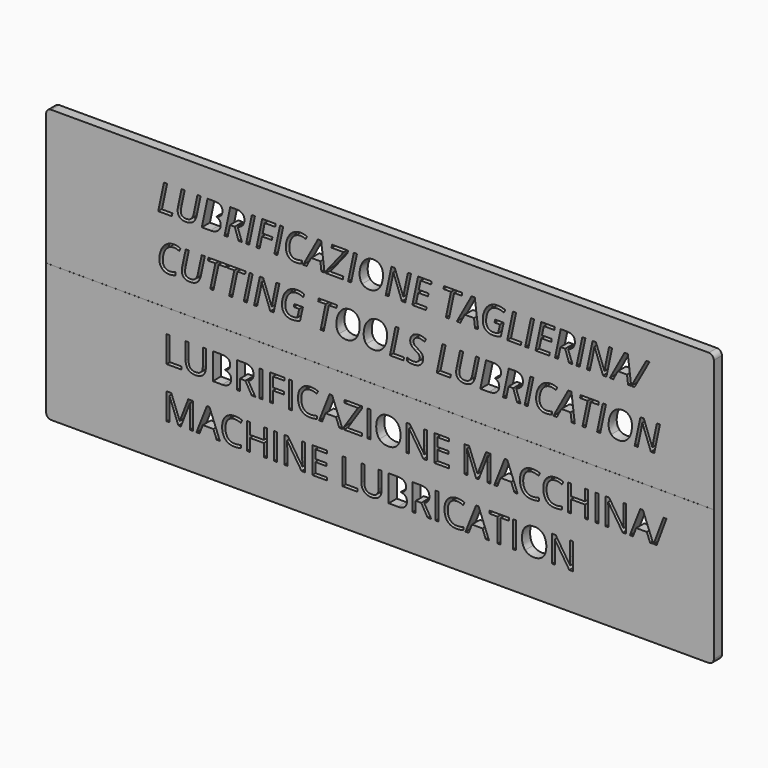
from build123d import *

# Parameters (mm, degrees)
F0_W     = 0.6068918224
F0_H     = 5.2220126864
F1_DEPTH = 2
F2_W     = 132
F2_H     = 0.01
F3_DEPTH = 0.01


with BuildPart() as f1:
    # F0 (on Front) → F1 (new body)
    with BuildSketch(Plane.XZ):
        with BuildLine():
            Line((-65, -27), (65, -27))
            ThreePointArc((65, -27), (65.7071067812, -26.7071067812), (66, -26))
            Line((66, -26), (66, 0))
            Line((66, 0), (-66, 0))
            Line((-66, 0), (-66, -26))
            ThreePointArc((-66, -26), (-65.7071067812, -26.7071067812), (-65, -27))
        make_face()
        with BuildLine():
            Line((-39.3672801544, -19.7942688532), (-39.8564509642, -19.7942688532))
            Line((-39.8564509642, -19.7942688532), (-41.6279807659, -15.1654329198))
            Line((-41.6279807659, -15.1654329198), (-41.6565538272, -15.1654329198))
            add(Edge.make_bspline(
                [(-41.6565538272, -15.1654329198), (-41.6062652393, -15.7151786195), (-41.6062652393, -16.4729362057)],
                knots=[0, 0, 0, 1, 1, 1], degree=2))
            Line((-41.6062652393, -16.4729362057), (-41.6062652393, -19.7942688532))
            Line((-41.6062652393, -19.7942688532), (-42.1674401636, -19.7942688532))
            Line((-42.1674401636, -19.7942688532), (-42.1674401636, -14.5722561668))
            Line((-42.1674401636, -14.5722561668), (-41.2531022014, -14.5722561668))
            Line((-41.2531022014, -14.5722561668), (-39.5992934123, -18.8799308911))
            Line((-39.5992934123, -18.8799308911), (-39.570720351, -18.8799308911))
            Line((-39.570720351, -18.8799308911), (-37.9031964925, -14.5722561668))
            Line((-37.9031964925, -14.5722561668), (-36.9957160651, -14.5722561668))
            Line((-36.9957160651, -14.5722561668), (-36.9957160651, -19.7942688532))
            Line((-36.9957160651, -19.7942688532), (-37.6026078875, -19.7942688532))
            Line((-37.6026078875, -19.7942688532), (-37.6026078875, -16.4295051525))
            add(Edge.make_bspline(
                [(-37.6026078875, -16.4295051525), (-37.6026078875, -15.8511863914), (-37.5523192995, -15.1722904545)],
                knots=[0, 0, 0, 1, 1, 1], degree=2))
            Line((-37.5523192995, -15.1722904545), (-37.5808923609, -15.1722904545))
            Line((-37.5808923609, -15.1722904545), (-39.3672801544, -19.7942688532))
        make_face(mode=Mode.SUBTRACT)
        Polygon((-31.6525535986, -19.7942688532), (-32.2811609476, -19.7942688532), (-32.9314838232, -18.1336025295), (-35.0241748341, -18.1336025295), (-35.6664972526, -19.7942688532), (-36.2813895321, -19.7942688532), (-34.2172715825, -14.5505406402), (-33.7063852462, -14.5505406402), align=None, mode=Mode.SUBTRACT)
        with BuildLine():
            add(Edge.make_bspline(
                [(-27.5128884749, -15.3185845284), (-28.1060652279, -15.0408543724), (-28.6992419808, -15.0408543724)],
                knots=[0, 0, 0, 1, 1, 1], degree=2))
            add(Edge.make_bspline(
                [(-28.6992419808, -15.0408543724), (-29.5598625877, -15.0408543724), (-30.0581767771, -15.6140299825)],
                knots=[0, 0, 0, 1, 1, 1], degree=2))
            add(Edge.make_bspline(
                [(-30.0581767771, -15.6140299825), (-30.5564909665, -16.1872055925), (-30.5564909665, -17.1838339713)],
                knots=[0, 0, 0, 1, 1, 1], degree=2))
            add(Edge.make_bspline(
                [(-30.5564909665, -17.1838339713), (-30.5564909665, -18.2078924889), (-30.0758920751, -18.7673530295)],
                knots=[0, 0, 0, 1, 1, 1], degree=2))
            add(Edge.make_bspline(
                [(-30.0758920751, -18.7673530295), (-29.5952931838, -19.3268135701), (-28.7060995156, -19.3268135701)],
                knots=[0, 0, 0, 1, 1, 1], degree=2))
            add(Edge.make_bspline(
                [(-28.7060995156, -19.3268135701), (-28.1597825832, -19.3268135701), (-27.4591711196, -19.1302309082)],
                knots=[0, 0, 0, 1, 1, 1], degree=2))
            Line((-27.4591711196, -19.1302309082), (-27.4591711196, -19.6616898487))
            add(Edge.make_bspline(
                [(-27.4591711196, -19.6616898487), (-28.0020592847, -19.8662729678), (-28.7986762342, -19.8662729678)],
                knots=[0, 0, 0, 1, 1, 1], degree=2))
            add(Edge.make_bspline(
                [(-28.7986762342, -19.8662729678), (-29.951884989, -19.8662729678), (-30.5787779543, -19.1656615043)],
                knots=[0, 0, 0, 1, 1, 1], degree=2))
            add(Edge.make_bspline(
                [(-30.5787779543, -19.1656615043), (-31.2056709196, -18.4650500407), (-31.2056709196, -17.1758335141)],
                knots=[0, 0, 0, 1, 1, 1], degree=2))
            add(Edge.make_bspline(
                [(-31.2056709196, -17.1758335141), (-31.2056709196, -16.3689302625), (-30.9039393921, -15.7620384401)],
                knots=[0, 0, 0, 1, 1, 1], degree=2))
            add(Edge.make_bspline(
                [(-30.9039393921, -15.7620384401), (-30.6022078646, -15.1551466177), (-30.0324610219, -14.8265564125)],
                knots=[0, 0, 0, 1, 1, 1], degree=2))
            add(Edge.make_bspline(
                [(-30.0324610219, -14.8265564125), (-29.4627141793, -14.4979662074), (-28.6912415237, -14.4979662074)],
                knots=[0, 0, 0, 1, 1, 1], degree=2))
            add(Edge.make_bspline(
                [(-28.6912415237, -14.4979662074), (-27.8706232026, -14.4979662074), (-27.2557309231, -14.79741189)],
                knots=[0, 0, 0, 1, 1, 1], degree=2))
            Line((-27.2557309231, -14.79741189), (-27.5128884749, -15.3185845284))
        make_face(mode=Mode.SUBTRACT)
        Polygon((-22.3548794458, -14.5722561668), (-22.3548794458, -19.7942688532), (-22.9617712682, -19.7942688532), (-22.9617712682, -17.3369855799), (-25.7127856119, -17.3369855799), (-25.7127856119, -19.7942688532), (-26.3196774343, -19.7942688532), (-26.3196774343, -14.5722561668), (-25.7127856119, -14.5722561668), (-25.7127856119, -16.7940974149), (-22.9617712682, -16.7940974149), (-22.9617712682, -14.5722561668), align=None, mode=Mode.SUBTRACT)
        with Locations((-20.6193517014, -17.18326251)):
            Rectangle(F0_W, F0_H, mode=Mode.SUBTRACT)
        with BuildLine():
            Line((-14.8047337232, -14.5722561668), (-14.8047337232, -19.7942688532))
            Line((-14.8047337232, -19.7942688532), (-15.4973447296, -19.7942688532))
            Line((-15.4973447296, -19.7942688532), (-18.351222094, -15.4123041696))
            Line((-18.351222094, -15.4123041696), (-18.3797951553, -15.4123041696))
            add(Edge.make_bspline(
                [(-18.3797951553, -15.4123041696), (-18.3226490327, -16.1837768251), (-18.3226490327, -16.8260992436)],
                knots=[0, 0, 0, 1, 1, 1], degree=2))
            Line((-18.3226490327, -16.8260992436), (-18.3226490327, -19.7942688532))
            Line((-18.3226490327, -19.7942688532), (-18.883823957, -19.7942688532))
            Line((-18.883823957, -19.7942688532), (-18.883823957, -14.5722561668))
            Line((-18.883823957, -14.5722561668), (-18.1980704853, -14.5722561668))
            Line((-18.1980704853, -14.5722561668), (-15.3510506556, -18.9370770137))
            Line((-15.3510506556, -18.9370770137), (-15.3224775943, -18.9370770137))
            add(Edge.make_bspline(
                [(-15.3224775943, -18.9370770137), (-15.329335129, -18.8410715277), (-15.354479423, -18.3176130443)],
                knots=[0, 0, 0, 1, 1, 1], degree=2))
            add(Edge.make_bspline(
                [(-15.354479423, -18.3176130443), (-15.3796237169, -17.794154561), (-15.3727661822, -17.5689988378)],
                knots=[0, 0, 0, 1, 1, 1], degree=2))
            Line((-15.3727661822, -17.5689988378), (-15.3727661822, -14.5722561668))
            Line((-15.3727661822, -14.5722561668), (-14.8047337232, -14.5722561668))
        make_face(mode=Mode.SUBTRACT)
        Polygon((-10.4581996356, -19.2513806882), (-10.4581996356, -19.7942688532), (-13.3692231226, -19.7942688532), (-13.3692231226, -14.5722561668), (-10.4581996356, -14.5722561668), (-10.4581996356, -15.1117155645), (-12.7623313002, -15.1117155645), (-12.7623313002, -16.7940974149), (-10.5976361748, -16.7940974149), (-10.5976361748, -17.3301280452), (-12.7623313002, -17.3301280452), (-12.7623313002, -19.2513806882), align=None, mode=Mode.SUBTRACT)
        Polygon((-4.4898585875, -19.7942688532), (-7.4008820746, -19.7942688532), (-7.4008820746, -14.5722561668), (-6.7939902522, -14.5722561668), (-6.7939902522, -19.2445231535), (-4.4898585875, -19.2445231535), align=None, mode=Mode.SUBTRACT)
        with BuildLine():
            Line((-0.2679030472, -14.5722561668), (0.3389887752, -14.5722561668))
            Line((0.3389887752, -14.5722561668), (0.3389887752, -17.950734937))
            add(Edge.make_bspline(
                [(0.3389887752, -17.950734937), (0.3389887752, -18.844500295), (-0.2004706225, -19.3553866314)],
                knots=[0, 0, 0, 1, 1, 1], degree=2))
            add(Edge.make_bspline(
                [(-0.2004706225, -19.3553866314), (-0.7399300202, -19.8662729678), (-1.6828410436, -19.8662729678)],
                knots=[0, 0, 0, 1, 1, 1], degree=2))
            add(Edge.make_bspline(
                [(-1.6828410436, -19.8662729678), (-2.6257520671, -19.8662729678), (-3.1417815545, -19.3513864028)],
                knots=[0, 0, 0, 1, 1, 1], degree=2))
            add(Edge.make_bspline(
                [(-3.1417815545, -19.3513864028), (-3.6578110419, -18.8364998379), (-3.6578110419, -17.9370198676)],
                knots=[0, 0, 0, 1, 1, 1], degree=2))
            Line((-3.6578110419, -17.9370198676), (-3.6578110419, -14.5722561668))
            Line((-3.6578110419, -14.5722561668), (-3.0497762971, -14.5722561668))
            Line((-3.0497762971, -14.5722561668), (-3.0497762971, -17.9793079983))
            add(Edge.make_bspline(
                [(-3.0497762971, -17.9793079983), (-3.0497762971, -18.6330596413), (-2.6926130306, -18.9833653731)],
                knots=[0, 0, 0, 1, 1, 1], degree=2))
            add(Edge.make_bspline(
                [(-2.6926130306, -18.9833653731), (-2.3354497641, -19.3336711048), (-1.6428387578, -19.3336711048)],
                knots=[0, 0, 0, 1, 1, 1], degree=2))
            add(Edge.make_bspline(
                [(-1.6428387578, -19.3336711048), (-0.9822295801, -19.3336711048), (-0.6250663137, -18.9816509894)],
                knots=[0, 0, 0, 1, 1, 1], degree=2))
            add(Edge.make_bspline(
                [(-0.6250663137, -18.9816509894), (-0.2679030472, -18.6296308739), (-0.2679030472, -17.9724504636)],
                knots=[0, 0, 0, 1, 1, 1], degree=2))
            Line((-0.2679030472, -17.9724504636), (-0.2679030472, -14.5722561668))
        make_face(mode=Mode.SUBTRACT)
        Polygon((-39.2564166765, -9.8462718248), (-42.1674401636, -9.8462718248), (-42.1674401636, -4.6242591384), (-41.5605483412, -4.6242591384), (-41.5605483412, -9.2965261251), (-39.2564166765, -9.2965261251), align=None, mode=Mode.SUBTRACT)
        with BuildLine():
            Line((-35.0344611362, -4.6242591384), (-34.4275693138, -4.6242591384))
            Line((-34.4275693138, -4.6242591384), (-34.4275693138, -8.0027379086))
            add(Edge.make_bspline(
                [(-34.4275693138, -8.0027379086), (-34.4275693138, -8.8965032666), (-34.9670287115, -9.407389603)],
                knots=[0, 0, 0, 1, 1, 1], degree=2))
            add(Edge.make_bspline(
                [(-34.9670287115, -9.407389603), (-35.5064881092, -9.9182759394), (-36.4493991327, -9.9182759394)],
                knots=[0, 0, 0, 1, 1, 1], degree=2))
            add(Edge.make_bspline(
                [(-36.4493991327, -9.9182759394), (-37.3923101562, -9.9182759394), (-37.9083396436, -9.4033893744)],
                knots=[0, 0, 0, 1, 1, 1], degree=2))
            add(Edge.make_bspline(
                [(-37.9083396436, -9.4033893744), (-38.424369131, -8.8885028095), (-38.424369131, -7.9890228392)],
                knots=[0, 0, 0, 1, 1, 1], degree=2))
            Line((-38.424369131, -7.9890228392), (-38.424369131, -4.6242591384))
            Line((-38.424369131, -4.6242591384), (-37.8163343861, -4.6242591384))
            Line((-37.8163343861, -4.6242591384), (-37.8163343861, -8.0313109699))
            add(Edge.make_bspline(
                [(-37.8163343861, -8.0313109699), (-37.8163343861, -8.6850626129), (-37.4591711196, -9.0353683446)],
                knots=[0, 0, 0, 1, 1, 1], degree=2))
            add(Edge.make_bspline(
                [(-37.4591711196, -9.0353683446), (-37.1020078532, -9.3856740764), (-36.4093968468, -9.3856740764)],
                knots=[0, 0, 0, 1, 1, 1], degree=2))
            add(Edge.make_bspline(
                [(-36.4093968468, -9.3856740764), (-35.7487876692, -9.3856740764), (-35.3916244027, -9.033653961)],
                knots=[0, 0, 0, 1, 1, 1], degree=2))
            add(Edge.make_bspline(
                [(-35.3916244027, -9.033653961), (-35.0344611362, -8.6816338455), (-35.0344611362, -8.0244534352)],
                knots=[0, 0, 0, 1, 1, 1], degree=2))
            Line((-35.0344611362, -8.0244534352), (-35.0344611362, -4.6242591384))
        make_face(mode=Mode.SUBTRACT)
        with BuildLine():
            Line((-33.0457760685, -9.8462718248), (-33.0457760685, -4.6242591384))
            Line((-33.0457760685, -4.6242591384), (-31.5702631821, -4.6242591384))
            add(Edge.make_bspline(
                [(-31.5702631821, -4.6242591384), (-30.5313466725, -4.6242591384), (-30.0667486955, -4.9351340455)],
                knots=[0, 0, 0, 1, 1, 1], degree=2))
            add(Edge.make_bspline(
                [(-30.0667486955, -4.9351340455), (-29.6021507185, -5.2460089527), (-29.6021507185, -5.9169044324)],
                knots=[0, 0, 0, 1, 1, 1], degree=2))
            add(Edge.make_bspline(
                [(-29.6021507185, -5.9169044324), (-29.6021507185, -6.3820738707), (-29.861022654, -6.6838053982)],
                knots=[0, 0, 0, 1, 1, 1], degree=2))
            add(Edge.make_bspline(
                [(-29.861022654, -6.6838053982), (-30.1198945896, -6.9855369257), (-30.6170658565, -7.074684877)],
                knots=[0, 0, 0, 1, 1, 1], degree=2))
            Line((-30.6170658565, -7.074684877), (-30.6170658565, -7.1101154731))
            add(Edge.make_bspline(
                [(-30.6170658565, -7.1101154731), (-29.4272835832, -7.3135556696), (-29.4272835832, -8.3604726363)],
                knots=[0, 0, 0, 1, 1, 1], degree=2))
            add(Edge.make_bspline(
                [(-29.4272835832, -8.3604726363), (-29.4272835832, -9.0599411774), (-29.9004534786, -9.4531065011)],
                knots=[0, 0, 0, 1, 1, 1], degree=2))
            add(Edge.make_bspline(
                [(-29.9004534786, -9.4531065011), (-30.3736233741, -9.8462718248), (-31.2239576789, -9.8462718248)],
                knots=[0, 0, 0, 1, 1, 1], degree=2))
            Line((-31.2239576789, -9.8462718248), (-33.0457760685, -9.8462718248))
        make_face(mode=Mode.SUBTRACT)
        with BuildLine():
            Line((-26.6088368148, -7.6747191647), (-27.6991848347, -7.6747191647))
            Line((-27.6991848347, -7.6747191647), (-27.6991848347, -9.8462718248))
            Line((-27.6991848347, -9.8462718248), (-28.3060766571, -9.8462718248))
            Line((-28.3060766571, -9.8462718248), (-28.3060766571, -4.6242591384))
            Line((-28.3060766571, -4.6242591384), (-26.8739948239, -4.6242591384))
            add(Edge.make_bspline(
                [(-26.8739948239, -4.6242591384), (-25.9127970411, -4.6242591384), (-25.4539136764, -4.9922801682)],
                knots=[0, 0, 0, 1, 1, 1], degree=2))
            add(Edge.make_bspline(
                [(-25.4539136764, -4.9922801682), (-24.9950303116, -5.360301198), (-24.9950303116, -6.0997720249)],
                knots=[0, 0, 0, 1, 1, 1], degree=2))
            add(Edge.make_bspline(
                [(-24.9950303116, -6.0997720249), (-24.9950303116, -7.135259767), (-26.0453760456, -7.4998520294)],
                knots=[0, 0, 0, 1, 1, 1], degree=2))
            Line((-26.0453760456, -7.4998520294), (-24.6270092818, -9.8462718248))
            Line((-24.6270092818, -9.8462718248), (-25.3447645821, -9.8462718248))
            Line((-25.3447645821, -9.8462718248), (-26.6088368148, -7.6747191647))
        make_face(mode=Mode.SUBTRACT)
        with Locations((-23.481229523, -7.2352654816)):
            Rectangle(F0_W, F0_H, mode=Mode.SUBTRACT)
        Polygon((-21.1388099562, -7.6141442747), (-21.1388099562, -9.8462718248), (-21.7457017785, -9.8462718248), (-21.7457017785, -4.6242591384), (-18.8346782915, -4.6242591384), (-18.8346782915, -5.1637185361), (-21.1388099562, -5.1637185361), (-21.1388099562, -7.074684877), (-18.9741148307, -7.074684877), (-18.9741148307, -7.6141442747), align=None, mode=Mode.SUBTRACT)
        with Locations((-17.667183006, -7.2352654816)):
            Rectangle(F0_W, F0_H, mode=Mode.SUBTRACT)
        with BuildLine():
            add(Edge.make_bspline(
                [(-12.5097454382, -5.3705875), (-13.1029221911, -5.092857344), (-13.6960989441, -5.092857344)],
                knots=[0, 0, 0, 1, 1, 1], degree=2))
            add(Edge.make_bspline(
                [(-13.6960989441, -5.092857344), (-14.556719551, -5.092857344), (-15.0550337404, -5.6660329541)],
                knots=[0, 0, 0, 1, 1, 1], degree=2))
            add(Edge.make_bspline(
                [(-15.0550337404, -5.6660329541), (-15.5533479298, -6.2392085641), (-15.5533479298, -7.2358369429)],
                knots=[0, 0, 0, 1, 1, 1], degree=2))
            add(Edge.make_bspline(
                [(-15.5533479298, -7.2358369429), (-15.5533479298, -8.2598954605), (-15.0727490384, -8.8193560011)],
                knots=[0, 0, 0, 1, 1, 1], degree=2))
            add(Edge.make_bspline(
                [(-15.0727490384, -8.8193560011), (-14.592150147, -9.3788165417), (-13.7029564788, -9.3788165417)],
                knots=[0, 0, 0, 1, 1, 1], degree=2))
            add(Edge.make_bspline(
                [(-13.7029564788, -9.3788165417), (-13.1566395464, -9.3788165417), (-12.4560280829, -9.1822338798)],
                knots=[0, 0, 0, 1, 1, 1], degree=2))
            Line((-12.4560280829, -9.1822338798), (-12.4560280829, -9.7136928203))
            add(Edge.make_bspline(
                [(-12.4560280829, -9.7136928203), (-12.9989162479, -9.9182759394), (-13.7955331975, -9.9182759394)],
                knots=[0, 0, 0, 1, 1, 1], degree=2))
            add(Edge.make_bspline(
                [(-13.7955331975, -9.9182759394), (-14.9487419523, -9.9182759394), (-15.5756349176, -9.2176644759)],
                knots=[0, 0, 0, 1, 1, 1], degree=2))
            add(Edge.make_bspline(
                [(-15.5756349176, -9.2176644759), (-16.2025278829, -8.5170530123), (-16.2025278829, -7.2278364857)],
                knots=[0, 0, 0, 1, 1, 1], degree=2))
            add(Edge.make_bspline(
                [(-16.2025278829, -7.2278364857), (-16.2025278829, -6.4209332341), (-15.9007963554, -5.8140414117)],
                knots=[0, 0, 0, 1, 1, 1], degree=2))
            add(Edge.make_bspline(
                [(-15.9007963554, -5.8140414117), (-15.5990648279, -5.2071495893), (-15.0293179852, -4.8785593841)],
                knots=[0, 0, 0, 1, 1, 1], degree=2))
            add(Edge.make_bspline(
                [(-15.0293179852, -4.8785593841), (-14.4595711425, -4.549969179), (-13.6880984869, -4.549969179)],
                knots=[0, 0, 0, 1, 1, 1], degree=2))
            add(Edge.make_bspline(
                [(-13.6880984869, -4.549969179), (-12.8674801659, -4.549969179), (-12.2525878863, -4.8494148616)],
                knots=[0, 0, 0, 1, 1, 1], degree=2))
            Line((-12.2525878863, -4.8494148616), (-12.5097454382, -5.3705875))
        make_face(mode=Mode.SUBTRACT)
        Polygon((-7.4054537644, -9.8462718248), (-8.0340611134, -9.8462718248), (-8.684383989, -8.1856055011), (-10.7770749999, -8.1856055011), (-11.4193974183, -9.8462718248), (-12.0342896979, -9.8462718248), (-9.9701717483, -4.6025436118), (-9.4592854119, -4.6025436118), align=None, mode=Mode.SUBTRACT)
        Polygon((-3.5229461925, -9.2965261251), (-3.5229461925, -9.8462718248), (-7.1128656165, -9.8462718248), (-7.1128656165, -9.3708160845), (-4.3412786687, -5.1705760708), (-7.0271464325, -5.1705760708), (-7.0271464325, -4.6242591384), (-3.6018078417, -4.6242591384), (-3.6018078417, -5.0997148787), (-6.3733947896, -9.2965261251), align=None, mode=Mode.SUBTRACT)
        with Locations((-2.2091568331, -7.2352654816)):
            Rectangle(F0_W, F0_H, mode=Mode.SUBTRACT)
        with BuildLine():
            Line((1.7207820205, -19.7942688532), (1.7207820205, -14.5722561668))
            Line((1.7207820205, -14.5722561668), (3.196294907, -14.5722561668))
            add(Edge.make_bspline(
                [(3.196294907, -14.5722561668), (4.2352114165, -14.5722561668), (4.6998093935, -14.8831310739)],
                knots=[0, 0, 0, 1, 1, 1], degree=2))
            add(Edge.make_bspline(
                [(4.6998093935, -14.8831310739), (5.1644073706, -15.1940059811), (5.1644073706, -15.8649014608)],
                knots=[0, 0, 0, 1, 1, 1], degree=2))
            add(Edge.make_bspline(
                [(5.1644073706, -15.8649014608), (5.1644073706, -16.3300708991), (4.905535435, -16.6318024266)],
                knots=[0, 0, 0, 1, 1, 1], degree=2))
            add(Edge.make_bspline(
                [(4.905535435, -16.6318024266), (4.6466634995, -16.9335339541), (4.1494922325, -17.0226819054)],
                knots=[0, 0, 0, 1, 1, 1], degree=2))
            Line((4.1494922325, -17.0226819054), (4.1494922325, -17.0581125015))
            add(Edge.make_bspline(
                [(4.1494922325, -17.0581125015), (5.3392745058, -17.261552698), (5.3392745058, -18.3084696647)],
                knots=[0, 0, 0, 1, 1, 1], degree=2))
            add(Edge.make_bspline(
                [(5.3392745058, -18.3084696647), (5.3392745058, -19.0079382058), (4.8661046104, -19.4011035295)],
                knots=[0, 0, 0, 1, 1, 1], degree=2))
            add(Edge.make_bspline(
                [(4.8661046104, -19.4011035295), (4.392934715, -19.7942688532), (3.5426004102, -19.7942688532)],
                knots=[0, 0, 0, 1, 1, 1], degree=2))
            Line((3.5426004102, -19.7942688532), (1.7207820205, -19.7942688532))
        make_face(mode=Mode.SUBTRACT)
        with BuildLine():
            Line((8.1577212742, -17.6227161931), (7.0673732543, -17.6227161931))
            Line((7.0673732543, -17.6227161931), (7.0673732543, -19.7942688532))
            Line((7.0673732543, -19.7942688532), (6.4604814319, -19.7942688532))
            Line((6.4604814319, -19.7942688532), (6.4604814319, -14.5722561668))
            Line((6.4604814319, -14.5722561668), (7.8925632652, -14.5722561668))
            add(Edge.make_bspline(
                [(7.8925632652, -14.5722561668), (8.8537610479, -14.5722561668), (9.3126444127, -14.9402771966)],
                knots=[0, 0, 0, 1, 1, 1], degree=2))
            add(Edge.make_bspline(
                [(9.3126444127, -14.9402771966), (9.7715277774, -15.3082982264), (9.7715277774, -16.0477690533)],
                knots=[0, 0, 0, 1, 1, 1], degree=2))
            add(Edge.make_bspline(
                [(9.7715277774, -16.0477690533), (9.7715277774, -17.0832567954), (8.7211820434, -17.4478490578)],
                knots=[0, 0, 0, 1, 1, 1], degree=2))
            Line((8.7211820434, -17.4478490578), (10.1395488072, -19.7942688532))
            Line((10.1395488072, -19.7942688532), (9.4217935069, -19.7942688532))
            Line((9.4217935069, -19.7942688532), (8.1577212742, -17.6227161931))
        make_face(mode=Mode.SUBTRACT)
        with Locations((11.285328566, -17.18326251)):
            Rectangle(F0_W, F0_H, mode=Mode.SUBTRACT)
        with BuildLine():
            add(Edge.make_bspline(
                [(16.4427661339, -15.3185845284), (15.849589381, -15.0408543724), (15.256412628, -15.0408543724)],
                knots=[0, 0, 0, 1, 1, 1], degree=2))
            add(Edge.make_bspline(
                [(15.256412628, -15.0408543724), (14.3957920211, -15.0408543724), (13.8974778317, -15.6140299825)],
                knots=[0, 0, 0, 1, 1, 1], degree=2))
            add(Edge.make_bspline(
                [(13.8974778317, -15.6140299825), (13.3991636423, -16.1872055925), (13.3991636423, -17.1838339713)],
                knots=[0, 0, 0, 1, 1, 1], degree=2))
            add(Edge.make_bspline(
                [(13.3991636423, -17.1838339713), (13.3991636423, -18.2078924889), (13.8797625337, -18.7673530295)],
                knots=[0, 0, 0, 1, 1, 1], degree=2))
            add(Edge.make_bspline(
                [(13.8797625337, -18.7673530295), (14.3603614251, -19.3268135701), (15.2495550933, -19.3268135701)],
                knots=[0, 0, 0, 1, 1, 1], degree=2))
            add(Edge.make_bspline(
                [(15.2495550933, -19.3268135701), (15.7958720257, -19.3268135701), (16.4964834892, -19.1302309082)],
                knots=[0, 0, 0, 1, 1, 1], degree=2))
            Line((16.4964834892, -19.1302309082), (16.4964834892, -19.6616898487))
            add(Edge.make_bspline(
                [(16.4964834892, -19.6616898487), (15.9535953241, -19.8662729678), (15.1569783746, -19.8662729678)],
                knots=[0, 0, 0, 1, 1, 1], degree=2))
            add(Edge.make_bspline(
                [(15.1569783746, -19.8662729678), (14.0037696198, -19.8662729678), (13.3768766545, -19.1656615043)],
                knots=[0, 0, 0, 1, 1, 1], degree=2))
            add(Edge.make_bspline(
                [(13.3768766545, -19.1656615043), (12.7499836892, -18.4650500407), (12.7499836892, -17.1758335141)],
                knots=[0, 0, 0, 1, 1, 1], degree=2))
            add(Edge.make_bspline(
                [(12.7499836892, -17.1758335141), (12.7499836892, -16.3689302625), (13.0517152167, -15.7620384401)],
                knots=[0, 0, 0, 1, 1, 1], degree=2))
            add(Edge.make_bspline(
                [(13.0517152167, -15.7620384401), (13.3534467442, -15.1551466177), (13.9231935869, -14.8265564125)],
                knots=[0, 0, 0, 1, 1, 1], degree=2))
            add(Edge.make_bspline(
                [(13.9231935869, -14.8265564125), (14.4929404296, -14.4979662074), (15.2644130852, -14.4979662074)],
                knots=[0, 0, 0, 1, 1, 1], degree=2))
            add(Edge.make_bspline(
                [(15.2644130852, -14.4979662074), (16.0850314062, -14.4979662074), (16.6999236858, -14.79741189)],
                knots=[0, 0, 0, 1, 1, 1], degree=2))
            Line((16.6999236858, -14.79741189), (16.4427661339, -15.3185845284))
        make_face(mode=Mode.SUBTRACT)
        Polygon((21.5470578077, -19.7942688532), (20.9184504587, -19.7942688532), (20.2681275831, -18.1336025295), (18.1754365722, -18.1336025295), (17.5331141538, -19.7942688532), (16.9182218742, -19.7942688532), (18.9823398238, -14.5505406402), (19.4932261602, -14.5505406402), align=None, mode=Mode.SUBTRACT)
        Polygon((23.8717620765, -15.1117155645), (23.8717620765, -19.7942688532), (23.2648702541, -19.7942688532), (23.2648702541, -15.1117155645), (21.6110614651, -15.1117155645), (21.6110614651, -14.5722561668), (25.5255708656, -14.5722561668), (25.5255708656, -15.1117155645), align=None, mode=Mode.SUBTRACT)
        with Locations((26.6153474243, -17.18326251)):
            Rectangle(F0_W, F0_H, mode=Mode.SUBTRACT)
        with BuildLine():
            add(Edge.make_bspline(
                [(32.2516694998, -15.2042922832), (32.8837056162, -15.9186188161), (32.8837056162, -17.1758335141)],
                knots=[0, 0, 0, 1, 1, 1], degree=2))
            add(Edge.make_bspline(
                [(32.8837056162, -17.1758335141), (32.8837056162, -18.4296194447), (32.2493836549, -19.1479462062)],
                knots=[0, 0, 0, 1, 1, 1], degree=2))
            add(Edge.make_bspline(
                [(32.2493836549, -19.1479462062), (31.6150616937, -19.8662729678), (30.4869972328, -19.8662729678)],
                knots=[0, 0, 0, 1, 1, 1], degree=2))
            add(Edge.make_bspline(
                [(30.4869972328, -19.8662729678), (29.333788478, -19.8662729678), (28.7068955127, -19.1605183532)],
                knots=[0, 0, 0, 1, 1, 1], degree=2))
            add(Edge.make_bspline(
                [(28.7068955127, -19.1605183532), (28.0800025474, -18.4547637387), (28.0800025474, -17.1689759794)],
                knots=[0, 0, 0, 1, 1, 1], degree=2))
            add(Edge.make_bspline(
                [(28.0800025474, -17.1689759794), (28.0800025474, -15.8934745221), (28.7086098964, -15.1917201362)],
                knots=[0, 0, 0, 1, 1, 1], degree=2))
            add(Edge.make_bspline(
                [(28.7086098964, -15.1917201362), (29.3372172454, -14.4899657502), (30.4938547675, -14.4899657502)],
                knots=[0, 0, 0, 1, 1, 1], degree=2))
            add(Edge.make_bspline(
                [(30.4938547675, -14.4899657502), (31.6196333835, -14.4899657502), (32.2516694998, -15.2042922832)],
                knots=[0, 0, 0, 1, 1, 1], degree=2))
        make_face(mode=Mode.SUBTRACT)
        with BuildLine():
            Line((38.1262909068, -14.5722561668), (38.1262909068, -19.7942688532))
            Line((38.1262909068, -19.7942688532), (37.4336799004, -19.7942688532))
            Line((37.4336799004, -19.7942688532), (34.579802536, -15.4123041696))
            Line((34.579802536, -15.4123041696), (34.5512294747, -15.4123041696))
            add(Edge.make_bspline(
                [(34.5512294747, -15.4123041696), (34.6083755973, -16.1837768251), (34.6083755973, -16.8260992436)],
                knots=[0, 0, 0, 1, 1, 1], degree=2))
            Line((34.6083755973, -16.8260992436), (34.6083755973, -19.7942688532))
            Line((34.6083755973, -19.7942688532), (34.047200673, -19.7942688532))
            Line((34.047200673, -19.7942688532), (34.047200673, -14.5722561668))
            Line((34.047200673, -14.5722561668), (34.7329541447, -14.5722561668))
            Line((34.7329541447, -14.5722561668), (37.5799739744, -18.9370770137))
            Line((37.5799739744, -18.9370770137), (37.6085470357, -18.9370770137))
            add(Edge.make_bspline(
                [(37.6085470357, -18.9370770137), (37.601689501, -18.8410715277), (37.576545207, -18.3176130443)],
                knots=[0, 0, 0, 1, 1, 1], degree=2))
            add(Edge.make_bspline(
                [(37.576545207, -18.3176130443), (37.551400913, -17.794154561), (37.5582584478, -17.5689988378)],
                knots=[0, 0, 0, 1, 1, 1], degree=2))
            Line((37.5582584478, -17.5689988378), (37.5582584478, -14.5722561668))
            Line((37.5582584478, -14.5722561668), (38.1262909068, -14.5722561668))
        make_face(mode=Mode.SUBTRACT)
        with BuildLine():
            add(Edge.make_bspline(
                [(3.4271652424, -5.2562952548), (4.0592013588, -5.9706217877), (4.0592013588, -7.2278364857)],
                knots=[0, 0, 0, 1, 1, 1], degree=2))
            add(Edge.make_bspline(
                [(4.0592013588, -7.2278364857), (4.0592013588, -8.4816224163), (3.4248793975, -9.1999491778)],
                knots=[0, 0, 0, 1, 1, 1], degree=2))
            add(Edge.make_bspline(
                [(3.4248793975, -9.1999491778), (2.7905574363, -9.9182759394), (1.6624929754, -9.9182759394)],
                knots=[0, 0, 0, 1, 1, 1], degree=2))
            add(Edge.make_bspline(
                [(1.6624929754, -9.9182759394), (0.5092842207, -9.9182759394), (-0.1176087447, -9.2125213248)],
                knots=[0, 0, 0, 1, 1, 1], degree=2))
            add(Edge.make_bspline(
                [(-0.1176087447, -9.2125213248), (-0.74450171, -8.5067667103), (-0.74450171, -7.220978951)],
                knots=[0, 0, 0, 1, 1, 1], degree=2))
            add(Edge.make_bspline(
                [(-0.74450171, -7.220978951), (-0.74450171, -5.9454774937), (-0.115894361, -5.2437231078)],
                knots=[0, 0, 0, 1, 1, 1], degree=2))
            add(Edge.make_bspline(
                [(-0.115894361, -5.2437231078), (0.512712988, -4.5419687218), (1.6693505102, -4.5419687218)],
                knots=[0, 0, 0, 1, 1, 1], degree=2))
            add(Edge.make_bspline(
                [(1.6693505102, -4.5419687218), (2.7951291261, -4.5419687218), (3.4271652424, -5.2562952548)],
                knots=[0, 0, 0, 1, 1, 1], degree=2))
        make_face(mode=Mode.SUBTRACT)
        with BuildLine():
            Line((9.3017866494, -4.6242591384), (9.3017866494, -9.8462718248))
            Line((9.3017866494, -9.8462718248), (8.609175643, -9.8462718248))
            Line((8.609175643, -9.8462718248), (5.7552982786, -5.4643071412))
            Line((5.7552982786, -5.4643071412), (5.7267252173, -5.4643071412))
            add(Edge.make_bspline(
                [(5.7267252173, -5.4643071412), (5.7838713399, -6.2357797967), (5.7838713399, -6.8781022152)],
                knots=[0, 0, 0, 1, 1, 1], degree=2))
            Line((5.7838713399, -6.8781022152), (5.7838713399, -9.8462718248))
            Line((5.7838713399, -9.8462718248), (5.2226964156, -9.8462718248))
            Line((5.2226964156, -9.8462718248), (5.2226964156, -4.6242591384))
            Line((5.2226964156, -4.6242591384), (5.9084498873, -4.6242591384))
            Line((5.9084498873, -4.6242591384), (8.755469717, -8.9890799853))
            Line((8.755469717, -8.9890799853), (8.7840427783, -8.9890799853))
            add(Edge.make_bspline(
                [(8.7840427783, -8.9890799853), (8.7771852436, -8.8930744993), (8.7520409496, -8.3696160159)],
                knots=[0, 0, 0, 1, 1, 1], degree=2))
            add(Edge.make_bspline(
                [(8.7520409496, -8.3696160159), (8.7268966557, -7.8461575326), (8.7337541904, -7.6210018094)],
                knots=[0, 0, 0, 1, 1, 1], degree=2))
            Line((8.7337541904, -7.6210018094), (8.7337541904, -4.6242591384))
            Line((8.7337541904, -4.6242591384), (9.3017866494, -4.6242591384))
        make_face(mode=Mode.SUBTRACT)
        Polygon((13.648320737, -9.3033836598), (13.648320737, -9.8462718248), (10.73729725, -9.8462718248), (10.73729725, -4.6242591384), (13.648320737, -4.6242591384), (13.648320737, -5.1637185361), (11.3441890724, -5.1637185361), (11.3441890724, -6.8461003865), (13.5088841978, -6.8461003865), (13.5088841978, -7.3821310168), (11.3441890724, -7.3821310168), (11.3441890724, -9.3033836598), align=None, mode=Mode.SUBTRACT)
        with BuildLine():
            Line((19.5057983072, -9.8462718248), (19.0166274974, -9.8462718248))
            Line((19.0166274974, -9.8462718248), (17.2450976957, -5.2174358914))
            Line((17.2450976957, -5.2174358914), (17.2165246344, -5.2174358914))
            add(Edge.make_bspline(
                [(17.2165246344, -5.2174358914), (17.2668132223, -5.7671815911), (17.2668132223, -6.5249391773)],
                knots=[0, 0, 0, 1, 1, 1], degree=2))
            Line((17.2668132223, -6.5249391773), (17.2668132223, -9.8462718248))
            Line((17.2668132223, -9.8462718248), (16.705638298, -9.8462718248))
            Line((16.705638298, -9.8462718248), (16.705638298, -4.6242591384))
            Line((16.705638298, -4.6242591384), (17.6199762602, -4.6242591384))
            Line((17.6199762602, -4.6242591384), (19.2737850493, -8.9319338627))
            Line((19.2737850493, -8.9319338627), (19.3023581106, -8.9319338627))
            Line((19.3023581106, -8.9319338627), (20.9698819691, -4.6242591384))
            Line((20.9698819691, -4.6242591384), (21.8773623966, -4.6242591384))
            Line((21.8773623966, -4.6242591384), (21.8773623966, -9.8462718248))
            Line((21.8773623966, -9.8462718248), (21.2704705742, -9.8462718248))
            Line((21.2704705742, -9.8462718248), (21.2704705742, -6.4815081241))
            add(Edge.make_bspline(
                [(21.2704705742, -6.4815081241), (21.2704705742, -5.903189363), (21.3207591621, -5.2242934261)],
                knots=[0, 0, 0, 1, 1, 1], degree=2))
            Line((21.3207591621, -5.2242934261), (21.2921861008, -5.2242934261))
            Line((21.2921861008, -5.2242934261), (19.5057983072, -9.8462718248))
        make_face(mode=Mode.SUBTRACT)
        Polygon((27.220524863, -9.8462718248), (26.591917514, -9.8462718248), (25.9415946384, -8.1856055011), (23.8489036275, -8.1856055011), (23.2065812091, -9.8462718248), (22.5916889295, -9.8462718248), (24.6558068791, -4.6025436118), (25.1666932155, -4.6025436118), align=None, mode=Mode.SUBTRACT)
        with BuildLine():
            add(Edge.make_bspline(
                [(31.3601899867, -5.3705875), (30.7670132337, -5.092857344), (30.1738364808, -5.092857344)],
                knots=[0, 0, 0, 1, 1, 1], degree=2))
            add(Edge.make_bspline(
                [(30.1738364808, -5.092857344), (29.3132158739, -5.092857344), (28.8149016845, -5.6660329541)],
                knots=[0, 0, 0, 1, 1, 1], degree=2))
            add(Edge.make_bspline(
                [(28.8149016845, -5.6660329541), (28.3165874951, -6.2392085641), (28.3165874951, -7.2358369429)],
                knots=[0, 0, 0, 1, 1, 1], degree=2))
            add(Edge.make_bspline(
                [(28.3165874951, -7.2358369429), (28.3165874951, -8.2598954605), (28.7971863865, -8.8193560011)],
                knots=[0, 0, 0, 1, 1, 1], degree=2))
            add(Edge.make_bspline(
                [(28.7971863865, -8.8193560011), (29.2777852779, -9.3788165417), (30.1669789461, -9.3788165417)],
                knots=[0, 0, 0, 1, 1, 1], degree=2))
            add(Edge.make_bspline(
                [(30.1669789461, -9.3788165417), (30.7132958785, -9.3788165417), (31.413907342, -9.1822338798)],
                knots=[0, 0, 0, 1, 1, 1], degree=2))
            Line((31.413907342, -9.1822338798), (31.413907342, -9.7136928203))
            add(Edge.make_bspline(
                [(31.413907342, -9.7136928203), (30.8710191769, -9.9182759394), (30.0744022274, -9.9182759394)],
                knots=[0, 0, 0, 1, 1, 1], degree=2))
            add(Edge.make_bspline(
                [(30.0744022274, -9.9182759394), (28.9211934726, -9.9182759394), (28.2943005073, -9.2176644759)],
                knots=[0, 0, 0, 1, 1, 1], degree=2))
            add(Edge.make_bspline(
                [(28.2943005073, -9.2176644759), (27.667407542, -8.5170530123), (27.667407542, -7.2278364857)],
                knots=[0, 0, 0, 1, 1, 1], degree=2))
            add(Edge.make_bspline(
                [(27.667407542, -7.2278364857), (27.667407542, -6.4209332341), (27.9691390695, -5.8140414117)],
                knots=[0, 0, 0, 1, 1, 1], degree=2))
            add(Edge.make_bspline(
                [(27.9691390695, -5.8140414117), (28.270870597, -5.2071495893), (28.8406174397, -4.8785593841)],
                knots=[0, 0, 0, 1, 1, 1], degree=2))
            add(Edge.make_bspline(
                [(28.8406174397, -4.8785593841), (29.4103642824, -4.549969179), (30.181836938, -4.549969179)],
                knots=[0, 0, 0, 1, 1, 1], degree=2))
            add(Edge.make_bspline(
                [(30.181836938, -4.549969179), (31.002455259, -4.549969179), (31.6173475386, -4.8494148616)],
                knots=[0, 0, 0, 1, 1, 1], degree=2))
            Line((31.6173475386, -4.8494148616), (31.3601899867, -5.3705875))
        make_face(mode=Mode.SUBTRACT)
        with BuildLine():
            add(Edge.make_bspline(
                [(35.9753108508, -5.3705875), (35.3821340978, -5.092857344), (34.7889573448, -5.092857344)],
                knots=[0, 0, 0, 1, 1, 1], degree=2))
            add(Edge.make_bspline(
                [(34.7889573448, -5.092857344), (33.9283367379, -5.092857344), (33.4300225486, -5.6660329541)],
                knots=[0, 0, 0, 1, 1, 1], degree=2))
            add(Edge.make_bspline(
                [(33.4300225486, -5.6660329541), (32.9317083592, -6.2392085641), (32.9317083592, -7.2358369429)],
                knots=[0, 0, 0, 1, 1, 1], degree=2))
            add(Edge.make_bspline(
                [(32.9317083592, -7.2358369429), (32.9317083592, -8.2598954605), (33.4123072505, -8.8193560011)],
                knots=[0, 0, 0, 1, 1, 1], degree=2))
            add(Edge.make_bspline(
                [(33.4123072505, -8.8193560011), (33.8929061419, -9.3788165417), (34.7820998101, -9.3788165417)],
                knots=[0, 0, 0, 1, 1, 1], degree=2))
            add(Edge.make_bspline(
                [(34.7820998101, -9.3788165417), (35.3284167425, -9.3788165417), (36.029028206, -9.1822338798)],
                knots=[0, 0, 0, 1, 1, 1], degree=2))
            Line((36.029028206, -9.1822338798), (36.029028206, -9.7136928203))
            add(Edge.make_bspline(
                [(36.029028206, -9.7136928203), (35.486140041, -9.9182759394), (34.6895230915, -9.9182759394)],
                knots=[0, 0, 0, 1, 1, 1], degree=2))
            add(Edge.make_bspline(
                [(34.6895230915, -9.9182759394), (33.5363143367, -9.9182759394), (32.9094213714, -9.2176644759)],
                knots=[0, 0, 0, 1, 1, 1], degree=2))
            add(Edge.make_bspline(
                [(32.9094213714, -9.2176644759), (32.282528406, -8.5170530123), (32.282528406, -7.2278364857)],
                knots=[0, 0, 0, 1, 1, 1], degree=2))
            add(Edge.make_bspline(
                [(32.282528406, -7.2278364857), (32.282528406, -6.4209332341), (32.5842599336, -5.8140414117)],
                knots=[0, 0, 0, 1, 1, 1], degree=2))
            add(Edge.make_bspline(
                [(32.5842599336, -5.8140414117), (32.8859914611, -5.2071495893), (33.4557383037, -4.8785593841)],
                knots=[0, 0, 0, 1, 1, 1], degree=2))
            add(Edge.make_bspline(
                [(33.4557383037, -4.8785593841), (34.0254851464, -4.549969179), (34.796957802, -4.549969179)],
                knots=[0, 0, 0, 1, 1, 1], degree=2))
            add(Edge.make_bspline(
                [(34.796957802, -4.549969179), (35.6175761231, -4.549969179), (36.2324684026, -4.8494148616)],
                knots=[0, 0, 0, 1, 1, 1], degree=2))
            Line((36.2324684026, -4.8494148616), (35.9753108508, -5.3705875))
        make_face(mode=Mode.SUBTRACT)
        Polygon((41.1333198798, -4.6242591384), (41.1333198798, -9.8462718248), (40.5264280574, -9.8462718248), (40.5264280574, -7.3889885515), (37.7754137138, -7.3889885515), (37.7754137138, -9.8462718248), (37.1685218914, -9.8462718248), (37.1685218914, -4.6242591384), (37.7754137138, -4.6242591384), (37.7754137138, -6.8461003865), (40.5264280574, -6.8461003865), (40.5264280574, -4.6242591384), align=None, mode=Mode.SUBTRACT)
        with Locations((42.8688476243, -7.2352654816)):
            Rectangle(F0_W, F0_H, mode=Mode.SUBTRACT)
        with BuildLine():
            Line((48.6834656025, -4.6242591384), (48.6834656025, -9.8462718248))
            Line((48.6834656025, -9.8462718248), (47.9908545961, -9.8462718248))
            Line((47.9908545961, -9.8462718248), (45.1369772317, -5.4643071412))
            Line((45.1369772317, -5.4643071412), (45.1084041704, -5.4643071412))
            add(Edge.make_bspline(
                [(45.1084041704, -5.4643071412), (45.165550293, -6.2357797967), (45.165550293, -6.8781022152)],
                knots=[0, 0, 0, 1, 1, 1], degree=2))
            Line((45.165550293, -6.8781022152), (45.165550293, -9.8462718248))
            Line((45.165550293, -9.8462718248), (44.6043753687, -9.8462718248))
            Line((44.6043753687, -9.8462718248), (44.6043753687, -4.6242591384))
            Line((44.6043753687, -4.6242591384), (45.2901288404, -4.6242591384))
            Line((45.2901288404, -4.6242591384), (48.1371486701, -8.9890799853))
            Line((48.1371486701, -8.9890799853), (48.1657217314, -8.9890799853))
            add(Edge.make_bspline(
                [(48.1657217314, -8.9890799853), (48.1588641967, -8.8930744993), (48.1337199027, -8.3696160159)],
                knots=[0, 0, 0, 1, 1, 1], degree=2))
            add(Edge.make_bspline(
                [(48.1337199027, -8.3696160159), (48.1085756087, -7.8461575326), (48.1154331435, -7.6210018094)],
                knots=[0, 0, 0, 1, 1, 1], degree=2))
            Line((48.1154331435, -7.6210018094), (48.1154331435, -4.6242591384))
            Line((48.1154331435, -4.6242591384), (48.6834656025, -4.6242591384))
        make_face(mode=Mode.SUBTRACT)
        Polygon((54.0300568362, -9.8462718248), (53.4014494872, -9.8462718248), (52.7511266117, -8.1856055011), (50.6584356007, -8.1856055011), (50.0161131823, -9.8462718248), (49.4012209028, -9.8462718248), (51.4653388524, -4.6025436118), (51.9762251887, -4.6025436118), align=None, mode=Mode.SUBTRACT)
        Polygon((56.0484578877, -4.6242591384), (56.6404917182, -4.6242591384), (54.6940947813, -9.8462718248), (54.1020609508, -9.8462718248), align=None, mode=Mode.SUBTRACT)
        with BuildLine():
            Line((-66, 0), (66, 0))
            Line((66, 0), (66, 26))
            ThreePointArc((66, 26), (65.7071067812, 26.7071067812), (65, 27))
            Line((65, 27), (-65, 27))
            ThreePointArc((-65, 27), (-65.7071067812, 26.7071067812), (-66, 26))
            Line((-66, 26), (-66, 0))
        make_face()
        with BuildLine():
            add(Edge.make_bspline(
                [(-39.6884145341, 10.6461235653), (-40.1945538161, 10.8980215876), (-40.7100660478, 10.8980215876)],
                knots=[0, 0, 0, 1, 1, 1], degree=2))
            add(Edge.make_bspline(
                [(-40.7100660478, 10.8980215876), (-41.3474266252, 10.8980215876), (-41.8506368604, 10.5430211189)],
                knots=[0, 0, 0, 1, 1, 1], degree=2))
            add(Edge.make_bspline(
                [(-41.8506368604, 10.5430211189), (-42.3538470957, 10.1880206503), (-42.6485092009, 9.5014520871)],
                knots=[0, 0, 0, 1, 1, 1], degree=2))
            add(Edge.make_bspline(
                [(-42.6485092009, 9.5014520871), (-42.943171306, 8.814883524), (-42.943171306, 8.0064666152)],
                knots=[0, 0, 0, 1, 1, 1], degree=2))
            add(Edge.make_bspline(
                [(-42.943171306, 8.0064666152), (-42.943171306, 7.3210696708), (-42.5864134093, 6.9127605509)],
                knots=[0, 0, 0, 1, 1, 1], degree=2))
            add(Edge.make_bspline(
                [(-42.5864134093, 6.9127605509), (-42.2296555126, 6.504451431), (-41.6040111223, 6.504451431)],
                knots=[0, 0, 0, 1, 1, 1], degree=2))
            add(Edge.make_bspline(
                [(-41.6040111223, 6.504451431), (-41.0943569842, 6.504451431), (-40.424191083, 6.7141711798)],
                knots=[0, 0, 0, 1, 1, 1], degree=2))
            Line((-40.424191083, 6.7141711798), (-40.424191083, 6.1681968617))
            add(Edge.make_bspline(
                [(-40.424191083, 6.1681968617), (-40.7393565155, 6.054549847), (-41.0252314804, 6.0029986238)],
                knots=[0, 0, 0, 1, 1, 1], degree=2))
            add(Edge.make_bspline(
                [(-41.0252314804, 6.0029986238), (-41.3111064452, 5.9514474007), (-41.7129716622, 5.9514474007)],
                knots=[0, 0, 0, 1, 1, 1], degree=2))
            add(Edge.make_bspline(
                [(-41.7129716622, 5.9514474007), (-42.5998870245, 5.9514474007), (-43.1048546878, 6.4991791469)],
                knots=[0, 0, 0, 1, 1, 1], degree=2))
            add(Edge.make_bspline(
                [(-43.1048546878, 6.4991791469), (-43.6098223511, 7.046910893), (-43.6098223511, 7.991235572)],
                knots=[0, 0, 0, 1, 1, 1], degree=2))
            add(Edge.make_bspline(
                [(-43.6098223511, 7.991235572), (-43.6098223511, 8.9472764381), (-43.2237739867, 9.769166962)],
                knots=[0, 0, 0, 1, 1, 1], degree=2))
            add(Edge.make_bspline(
                [(-43.2237739867, 9.769166962), (-42.8377256223, 10.591057486), (-42.185719811, 11.02279898)],
                knots=[0, 0, 0, 1, 1, 1], degree=2))
            add(Edge.make_bspline(
                [(-42.185719811, 11.02279898), (-41.5337139998, 11.4545404741), (-40.7100660478, 11.4545404741)],
                knots=[0, 0, 0, 1, 1, 1], degree=2))
            add(Edge.make_bspline(
                [(-40.7100660478, 11.4545404741), (-39.9895205421, 11.4545404741), (-39.4365165118, 11.161635797)],
                knots=[0, 0, 0, 1, 1, 1], degree=2))
            Line((-39.4365165118, 11.161635797), (-39.6884145341, 10.6461235653))
        make_face(mode=Mode.SUBTRACT)
        with BuildLine():
            Line((-35.2432931544, 11.378385258), (-34.6211636202, 11.378385258))
            Line((-34.6211636202, 11.378385258), (-35.3721712123, 7.8412683773))
            add(Edge.make_bspline(
                [(-35.3721712123, 7.8412683773), (-35.5736896301, 6.878197799), (-36.0950599554, 6.4148225998)],
                knots=[0, 0, 0, 1, 1, 1], degree=2))
            add(Edge.make_bspline(
                [(-36.0950599554, 6.4148225998), (-36.6164302806, 5.9514474007), (-37.5174050674, 5.9514474007)],
                knots=[0, 0, 0, 1, 1, 1], degree=2))
            add(Edge.make_bspline(
                [(-37.5174050674, 5.9514474007), (-38.3597989187, 5.9514474007), (-38.7657648012, 6.3328092903)],
                knots=[0, 0, 0, 1, 1, 1], degree=2))
            add(Edge.make_bspline(
                [(-38.7657648012, 6.3328092903), (-39.1717306837, 6.7141711798), (-39.1717306837, 7.4276869733)],
                knots=[0, 0, 0, 1, 1, 1], degree=2))
            add(Edge.make_bspline(
                [(-39.1717306837, 7.4276869733), (-39.1717306837, 7.7241065065), (-39.0838592805, 8.1634635221)],
                knots=[0, 0, 0, 1, 1, 1], degree=2))
            Line((-39.0838592805, 8.1634635221), (-38.3926042426, 11.378385258))
            Line((-38.3926042426, 11.378385258), (-37.7704747084, 11.378385258))
            Line((-37.7704747084, 11.378385258), (-38.4687594586, 8.1154271551))
            add(Edge.make_bspline(
                [(-38.4687594586, 8.1154271551), (-38.5496011495, 7.7276213626), (-38.5496011495, 7.4276869733)],
                knots=[0, 0, 0, 1, 1, 1], degree=2))
            add(Edge.make_bspline(
                [(-38.5496011495, 7.4276869733), (-38.5496011495, 6.998874526), (-38.282472084, 6.7516629785)],
                knots=[0, 0, 0, 1, 1, 1], degree=2))
            add(Edge.make_bspline(
                [(-38.282472084, 6.7516629785), (-38.0153430185, 6.504451431), (-37.4845997436, 6.504451431)],
                knots=[0, 0, 0, 1, 1, 1], degree=2))
            add(Edge.make_bspline(
                [(-37.4845997436, 6.504451431), (-36.8542688784, 6.504451431), (-36.504540694, 6.8248891478)],
                knots=[0, 0, 0, 1, 1, 1], degree=2))
            add(Edge.make_bspline(
                [(-36.504540694, 6.8248891478), (-36.1548125095, 7.1453268645), (-35.9943007465, 7.8857898883)],
                knots=[0, 0, 0, 1, 1, 1], degree=2))
            Line((-35.9943007465, 7.8857898883), (-35.2432931544, 11.378385258))
        make_face(mode=Mode.SUBTRACT)
        Polygon((-31.9006649793, 10.8253812276), (-32.922316493, 6.0252593793), (-33.5526473581, 6.0252593793), (-32.5380255567, 10.8253812276), (-34.0248096976, 10.8253812276), (-33.9041329707, 11.378385258), (-30.2967189675, 11.378385258), (-30.4068511261, 10.8253812276), align=None, mode=Mode.SUBTRACT)
        Polygon((-28.1655445369, 10.8253812276), (-29.1871960506, 6.0252593793), (-29.8175269157, 6.0252593793), (-28.8029051143, 10.8253812276), (-30.2896892552, 10.8253812276), (-30.1690125283, 11.378385258), (-26.5615985251, 11.378385258), (-26.6717306837, 10.8253812276), align=None, mode=Mode.SUBTRACT)
        Polygon((-26.3050140279, 6.0252593793), (-26.9201138498, 6.0252593793), (-25.7813004653, 11.378385258), (-25.1662006434, 11.378385258), align=None, mode=Mode.SUBTRACT)
        with BuildLine():
            Line((-19.8868867433, 11.378385258), (-21.0186704156, 6.0252593793))
            Line((-21.0186704156, 6.0252593793), (-21.6806349858, 6.0252593793))
            Line((-21.6806349858, 6.0252593793), (-23.3654226885, 10.5031860828))
            Line((-23.3654226885, 10.5031860828), (-23.3865118253, 10.5031860828))
            add(Edge.make_bspline(
                [(-23.3865118253, 10.5031860828), (-23.5036736961, 9.6935975553), (-23.6583273656, 8.9730520497)],
                knots=[0, 0, 0, 1, 1, 1], degree=2))
            Line((-23.6583273656, 8.9730520497), (-24.2874866121, 6.0252593793))
            Line((-24.2874866121, 6.0252593793), (-24.8803256785, 6.0252593793))
            Line((-24.8803256785, 6.0252593793), (-23.7497136249, 11.378385258))
            Line((-23.7497136249, 11.378385258), (-23.0900922921, 11.378385258))
            Line((-23.0900922921, 11.378385258), (-21.4099910642, 6.9110031229))
            Line((-21.4099910642, 6.9110031229), (-21.3877303087, 6.9110031229))
            add(Edge.make_bspline(
                [(-21.3877303087, 6.9110031229), (-21.2775981502, 7.7311362187), (-21.1241160994, 8.3942724077)],
                knots=[0, 0, 0, 1, 1, 1], degree=2))
            Line((-21.1241160994, 8.3942724077), (-20.486755522, 11.378385258))
            Line((-20.486755522, 11.378385258), (-19.8868867433, 11.378385258))
        make_face(mode=Mode.SUBTRACT)
        with BuildLine():
            Line((-17.0375100444, 8.2735956807), (-16.9168333175, 8.8301145672))
            Line((-16.9168333175, 8.8301145672), (-15.2367320896, 8.8301145672))
            Line((-15.2367320896, 8.8301145672), (-15.8002806884, 6.2267777971))
            add(Edge.make_bspline(
                [(-15.8002806884, 6.2267777971), (-16.5911233165, 5.9514474007), (-17.3351011964, 5.9514474007)],
                knots=[0, 0, 0, 1, 1, 1], degree=2))
            add(Edge.make_bspline(
                [(-17.3351011964, 5.9514474007), (-18.3016866308, 5.9514474007), (-18.8377021899, 6.4810190569)],
                knots=[0, 0, 0, 1, 1, 1], degree=2))
            add(Edge.make_bspline(
                [(-18.8377021899, 6.4810190569), (-19.373717749, 7.0105907131), (-19.373717749, 7.9584302482)],
                knots=[0, 0, 0, 1, 1, 1], degree=2))
            add(Edge.make_bspline(
                [(-19.373717749, 7.9584302482), (-19.373717749, 8.9437615819), (-19.0023146184, 9.751006872)],
                knots=[0, 0, 0, 1, 1, 1], degree=2))
            add(Edge.make_bspline(
                [(-19.0023146184, 9.751006872), (-18.6309114879, 10.5582521621), (-17.9718759644, 11.0063963181)],
                knots=[0, 0, 0, 1, 1, 1], degree=2))
            add(Edge.make_bspline(
                [(-17.9718759644, 11.0063963181), (-17.3128404409, 11.4545404741), (-16.5102816256, 11.4545404741)],
                knots=[0, 0, 0, 1, 1, 1], degree=2))
            add(Edge.make_bspline(
                [(-16.5102816256, 11.4545404741), (-16.0826407971, 11.4545404741), (-15.707137001, 11.3813143048)],
                knots=[0, 0, 0, 1, 1, 1], degree=2))
            add(Edge.make_bspline(
                [(-15.707137001, 11.3813143048), (-15.331633205, 11.3080881355), (-14.9508571248, 11.1475763725)],
                knots=[0, 0, 0, 1, 1, 1], degree=2))
            Line((-14.9508571248, 11.1475763725), (-15.1922105787, 10.591057486))
            add(Edge.make_bspline(
                [(-15.1922105787, 10.591057486), (-15.4745706874, 10.7152490691), (-15.7985232603, 10.8066353283)],
                knots=[0, 0, 0, 1, 1, 1], degree=2))
            add(Edge.make_bspline(
                [(-15.7985232603, 10.8066353283), (-16.1224758332, 10.8980215876), (-16.5102816256, 10.8980215876)],
                knots=[0, 0, 0, 1, 1, 1], degree=2))
            add(Edge.make_bspline(
                [(-16.5102816256, 10.8980215876), (-17.1300679224, 10.8980215876), (-17.6367930138, 10.526618457)],
                knots=[0, 0, 0, 1, 1, 1], degree=2))
            add(Edge.make_bspline(
                [(-17.6367930138, 10.526618457), (-18.1435181052, 10.1552153264), (-18.4252924045, 9.4891500907)],
                knots=[0, 0, 0, 1, 1, 1], degree=2))
            add(Edge.make_bspline(
                [(-18.4252924045, 9.4891500907), (-18.7070667039, 8.823084855), (-18.7070667039, 7.9982652843)],
                knots=[0, 0, 0, 1, 1, 1], degree=2))
            add(Edge.make_bspline(
                [(-18.7070667039, 7.9982652843), (-18.7070667039, 7.3034953902), (-18.3321487172, 6.9039734106)],
                knots=[0, 0, 0, 1, 1, 1], degree=2))
            add(Edge.make_bspline(
                [(-18.3321487172, 6.9039734106), (-17.9572307305, 6.504451431), (-17.2835499732, 6.504451431)],
                knots=[0, 0, 0, 1, 1, 1], degree=2))
            add(Edge.make_bspline(
                [(-17.2835499732, 6.504451431), (-16.7200013745, 6.504451431), (-16.3310239633, 6.6473889135)],
                knots=[0, 0, 0, 1, 1, 1], degree=2))
            Line((-16.3310239633, 6.6473889135), (-15.9795383507, 8.2735956807))
            Line((-15.9795383507, 8.2735956807), (-17.0375100444, 8.2735956807))
        make_face(mode=Mode.SUBTRACT)
        Polygon((-10.0956691971, 10.8253812276), (-11.1173207108, 6.0252593793), (-11.747651576, 6.0252593793), (-10.7330297745, 10.8253812276), (-12.2198139155, 10.8253812276), (-12.0991371885, 11.378385258), (-8.4917231853, 11.378385258), (-8.6018553439, 10.8253812276), align=None, mode=Mode.SUBTRACT)
        with BuildLine():
            add(Edge.make_bspline(
                [(-4.5123202422, 10.8986073969), (-3.9997370573, 10.3344729888), (-3.9997370573, 9.3456267989)],
                knots=[0, 0, 0, 1, 1, 1], degree=2))
            add(Edge.make_bspline(
                [(-3.9997370573, 9.3456267989), (-3.9997370573, 8.3614670839), (-4.3219322021, 7.5835122615)],
                knots=[0, 0, 0, 1, 1, 1], degree=2))
            add(Edge.make_bspline(
                [(-4.3219322021, 7.5835122615), (-4.6441273469, 6.8055574391), (-5.244581935, 6.3785024199)],
                knots=[0, 0, 0, 1, 1, 1], degree=2))
            add(Edge.make_bspline(
                [(-5.244581935, 6.3785024199), (-5.845036523, 5.9514474007), (-6.6311926764, 5.9514474007)],
                knots=[0, 0, 0, 1, 1, 1], degree=2))
            add(Edge.make_bspline(
                [(-6.6311926764, 5.9514474007), (-7.5684876431, 5.9514474007), (-8.0922012057, 6.4991791469)],
                knots=[0, 0, 0, 1, 1, 1], degree=2))
            add(Edge.make_bspline(
                [(-8.0922012057, 6.4991791469), (-8.6159147684, 7.046910893), (-8.6159147684, 8.0357570829)],
                knots=[0, 0, 0, 1, 1, 1], degree=2))
            add(Edge.make_bspline(
                [(-8.6159147684, 8.0357570829), (-8.6159147684, 9.0023425174), (-8.2644291559, 9.8002148578)],
                knots=[0, 0, 0, 1, 1, 1], degree=2))
            add(Edge.make_bspline(
                [(-8.2644291559, 9.8002148578), (-7.9129435434, 10.5980871982), (-7.2996011495, 11.0304145016)],
                knots=[0, 0, 0, 1, 1, 1], degree=2))
            add(Edge.make_bspline(
                [(-7.2996011495, 11.0304145016), (-6.6862587556, 11.462741805), (-5.9176768829, 11.462741805)],
                knots=[0, 0, 0, 1, 1, 1], degree=2))
            add(Edge.make_bspline(
                [(-5.9176768829, 11.462741805), (-5.0249034271, 11.462741805), (-4.5123202422, 10.8986073969)],
                knots=[0, 0, 0, 1, 1, 1], degree=2))
        make_face(mode=Mode.SUBTRACT)
        with BuildLine():
            add(Edge.make_bspline(
                [(0.8876703849, 10.8986073969), (1.4002535698, 10.3344729888), (1.4002535698, 9.3456267989)],
                knots=[0, 0, 0, 1, 1, 1], degree=2))
            add(Edge.make_bspline(
                [(1.4002535698, 9.3456267989), (1.4002535698, 8.3614670839), (1.078058425, 7.5835122615)],
                knots=[0, 0, 0, 1, 1, 1], degree=2))
            add(Edge.make_bspline(
                [(1.078058425, 7.5835122615), (0.7558632802, 6.8055574391), (0.1554086921, 6.3785024199)],
                knots=[0, 0, 0, 1, 1, 1], degree=2))
            add(Edge.make_bspline(
                [(0.1554086921, 6.3785024199), (-0.445045896, 5.9514474007), (-1.2312020493, 5.9514474007)],
                knots=[0, 0, 0, 1, 1, 1], degree=2))
            add(Edge.make_bspline(
                [(-1.2312020493, 5.9514474007), (-2.168497016, 5.9514474007), (-2.6922105787, 6.4991791469)],
                knots=[0, 0, 0, 1, 1, 1], degree=2))
            add(Edge.make_bspline(
                [(-2.6922105787, 6.4991791469), (-3.2159241413, 7.046910893), (-3.2159241413, 8.0357570829)],
                knots=[0, 0, 0, 1, 1, 1], degree=2))
            add(Edge.make_bspline(
                [(-3.2159241413, 8.0357570829), (-3.2159241413, 9.0023425174), (-2.8644385288, 9.8002148578)],
                knots=[0, 0, 0, 1, 1, 1], degree=2))
            add(Edge.make_bspline(
                [(-2.8644385288, 9.8002148578), (-2.5129529163, 10.5980871982), (-1.8996105224, 11.0304145016)],
                knots=[0, 0, 0, 1, 1, 1], degree=2))
            add(Edge.make_bspline(
                [(-1.8996105224, 11.0304145016), (-1.2862681286, 11.462741805), (-0.5176862559, 11.462741805)],
                knots=[0, 0, 0, 1, 1, 1], degree=2))
            add(Edge.make_bspline(
                [(-0.5176862559, 11.462741805), (0.3750871999, 11.462741805), (0.8876703849, 10.8986073969)],
                knots=[0, 0, 0, 1, 1, 1], degree=2))
        make_face(mode=Mode.SUBTRACT)
        Polygon((-41.1529379196, 16.2230286173), (-43.8441460928, 16.2230286173), (-42.7135340392, 21.576154496), (-42.0902328863, 21.576154496), (-43.1013398317, 16.786577216), (-41.0322611926, 16.786577216), align=None, mode=Mode.SUBTRACT)
        with BuildLine():
            Line((-36.0751424373, 21.576154496), (-35.4530129032, 21.576154496))
            Line((-35.4530129032, 21.576154496), (-36.2040204953, 18.0390376153))
            add(Edge.make_bspline(
                [(-36.2040204953, 18.0390376153), (-36.4055389131, 17.075967037), (-36.9269092384, 16.6125918378)],
                knots=[0, 0, 0, 1, 1, 1], degree=2))
            add(Edge.make_bspline(
                [(-36.9269092384, 16.6125918378), (-37.4482795636, 16.1492166387), (-38.3492543504, 16.1492166387)],
                knots=[0, 0, 0, 1, 1, 1], degree=2))
            add(Edge.make_bspline(
                [(-38.3492543504, 16.1492166387), (-39.1916482017, 16.1492166387), (-39.5976140842, 16.5305785282)],
                knots=[0, 0, 0, 1, 1, 1], degree=2))
            add(Edge.make_bspline(
                [(-39.5976140842, 16.5305785282), (-40.0035799666, 16.9119404178), (-40.0035799666, 17.6254562112)],
                knots=[0, 0, 0, 1, 1, 1], degree=2))
            add(Edge.make_bspline(
                [(-40.0035799666, 17.6254562112), (-40.0035799666, 17.9218757445), (-39.9157085635, 18.3612327601)],
                knots=[0, 0, 0, 1, 1, 1], degree=2))
            Line((-39.9157085635, 18.3612327601), (-39.2244535255, 21.576154496))
            Line((-39.2244535255, 21.576154496), (-38.6023239914, 21.576154496))
            Line((-38.6023239914, 21.576154496), (-39.3006087416, 18.3131963931))
            add(Edge.make_bspline(
                [(-39.3006087416, 18.3131963931), (-39.3814504325, 17.9253906006), (-39.3814504325, 17.6254562112)],
                knots=[0, 0, 0, 1, 1, 1], degree=2))
            add(Edge.make_bspline(
                [(-39.3814504325, 17.6254562112), (-39.3814504325, 17.196643764), (-39.114321367, 16.9494322165)],
                knots=[0, 0, 0, 1, 1, 1], degree=2))
            add(Edge.make_bspline(
                [(-39.114321367, 16.9494322165), (-38.8471923014, 16.702220669), (-38.3164490265, 16.702220669)],
                knots=[0, 0, 0, 1, 1, 1], degree=2))
            add(Edge.make_bspline(
                [(-38.3164490265, 16.702220669), (-37.6861181614, 16.702220669), (-37.3363899769, 17.0226583858)],
                knots=[0, 0, 0, 1, 1, 1], degree=2))
            add(Edge.make_bspline(
                [(-37.3363899769, 17.0226583858), (-36.9866617925, 17.3430961025), (-36.8261500294, 18.0835591262)],
                knots=[0, 0, 0, 1, 1, 1], degree=2))
            Line((-36.8261500294, 18.0835591262), (-36.0751424373, 21.576154496))
        make_face(mode=Mode.SUBTRACT)
        with BuildLine():
            Line((-34.091591964, 21.576154496), (-32.7184548378, 21.576154496))
            add(Edge.make_bspline(
                [(-32.7184548378, 21.576154496), (-31.1367695814, 21.576154496), (-31.1367695814, 20.3459548522)],
                knots=[0, 0, 0, 1, 1, 1], degree=2))
            add(Edge.make_bspline(
                [(-31.1367695814, 20.3459548522), (-31.1367695814, 19.8292710018), (-31.4548640607, 19.4742705331)],
                knots=[0, 0, 0, 1, 1, 1], degree=2))
            add(Edge.make_bspline(
                [(-31.4548640607, 19.4742705331), (-31.7729585401, 19.1192700645), (-32.351738182, 19.012652762)],
                knots=[0, 0, 0, 1, 1, 1], degree=2))
            Line((-32.351738182, 19.012652762), (-32.351738182, 18.976332582))
            add(Edge.make_bspline(
                [(-32.351738182, 18.976332582), (-31.9311270657, 18.8591707112), (-31.7055904643, 18.5715383183)],
                knots=[0, 0, 0, 1, 1, 1], degree=2))
            add(Edge.make_bspline(
                [(-31.7055904643, 18.5715383183), (-31.480053863, 18.2839059254), (-31.480053863, 17.8820407084)],
                knots=[0, 0, 0, 1, 1, 1], degree=2))
            add(Edge.make_bspline(
                [(-31.480053863, 17.8820407084), (-31.480053863, 17.1052575047), (-32.0365727495, 16.664143061)],
                knots=[0, 0, 0, 1, 1, 1], degree=2))
            add(Edge.make_bspline(
                [(-32.0365727495, 16.664143061), (-32.593091636, 16.2230286173), (-33.5268717466, 16.2230286173)],
                knots=[0, 0, 0, 1, 1, 1], degree=2))
            Line((-33.5268717466, 16.2230286173), (-35.2222040176, 16.2230286173))
            Line((-35.2222040176, 16.2230286173), (-34.091591964, 21.576154496))
        make_face(mode=Mode.SUBTRACT)
        with BuildLine():
            Line((-28.719720186, 18.4491041633), (-29.6429557282, 18.4491041633))
            Line((-29.6429557282, 18.4491041633), (-30.1151180677, 16.2230286173))
            Line((-30.1151180677, 16.2230286173), (-30.7372476018, 16.2230286173))
            Line((-30.7372476018, 16.2230286173), (-29.6066355482, 21.576154496))
            Line((-29.6066355482, 21.576154496), (-28.4350168398, 21.576154496))
            add(Edge.make_bspline(
                [(-28.4350168398, 21.576154496), (-26.8017803603, 21.576154496), (-26.8017803603, 20.2358226936)],
                knots=[0, 0, 0, 1, 1, 1], degree=2))
            add(Edge.make_bspline(
                [(-26.8017803603, 20.2358226936), (-26.8017803603, 18.9622731575), (-28.149141875, 18.5920416457)],
                knots=[0, 0, 0, 1, 1, 1], degree=2))
            Line((-28.149141875, 18.5920416457), (-27.2739426998, 16.2230286173))
            Line((-27.2739426998, 16.2230286173), (-27.9546531694, 16.2230286173))
            Line((-27.9546531694, 16.2230286173), (-28.719720186, 18.4491041633))
        make_face(mode=Mode.SUBTRACT)
        Polygon((-25.8562840626, 16.2230286173), (-26.4713838845, 16.2230286173), (-25.3325705, 21.576154496), (-24.717470678, 21.576154496), align=None, mode=Mode.SUBTRACT)
        Polygon((-23.3150430841, 18.5041702425), (-23.7954067545, 16.2230286173), (-24.4245660009, 16.2230286173), (-23.2939539473, 21.576154496), (-20.6027457741, 21.576154496), (-20.711706314, 21.0161207534), (-22.7913295214, 21.0161207534), (-23.1943663571, 19.0642039852), (-21.2611954882, 19.0642039852), (-21.3783573591, 18.5041702425), align=None, mode=Mode.SUBTRACT)
        Polygon((-20.2688344422, 16.2230286173), (-20.8839342641, 16.2230286173), (-19.7451208796, 21.576154496), (-19.1300210576, 21.576154496), align=None, mode=Mode.SUBTRACT)
        with BuildLine():
            add(Edge.make_bspline(
                [(-14.6813848218, 20.8438928032), (-15.1875241039, 21.0957908255), (-15.7030363356, 21.0957908255)],
                knots=[0, 0, 0, 1, 1, 1], degree=2))
            add(Edge.make_bspline(
                [(-15.7030363356, 21.0957908255), (-16.3403969129, 21.0957908255), (-16.8436071482, 20.7407903569)],
                knots=[0, 0, 0, 1, 1, 1], degree=2))
            add(Edge.make_bspline(
                [(-16.8436071482, 20.7407903569), (-17.3468173834, 20.3857898883), (-17.6414794886, 19.6992213251)],
                knots=[0, 0, 0, 1, 1, 1], degree=2))
            add(Edge.make_bspline(
                [(-17.6414794886, 19.6992213251), (-17.9361415938, 19.012652762), (-17.9361415938, 18.2042358532)],
                knots=[0, 0, 0, 1, 1, 1], degree=2))
            add(Edge.make_bspline(
                [(-17.9361415938, 18.2042358532), (-17.9361415938, 17.5188389088), (-17.5793836971, 17.1105297889)],
                knots=[0, 0, 0, 1, 1, 1], degree=2))
            add(Edge.make_bspline(
                [(-17.5793836971, 17.1105297889), (-17.2226258004, 16.702220669), (-16.5969814101, 16.702220669)],
                knots=[0, 0, 0, 1, 1, 1], degree=2))
            add(Edge.make_bspline(
                [(-16.5969814101, 16.702220669), (-16.0873272719, 16.702220669), (-15.4171613707, 16.9119404178)],
                knots=[0, 0, 0, 1, 1, 1], degree=2))
            Line((-15.4171613707, 16.9119404178), (-15.4171613707, 16.3659660997))
            add(Edge.make_bspline(
                [(-15.4171613707, 16.3659660997), (-15.7323268033, 16.252319085), (-16.0182017681, 16.2007678618)],
                knots=[0, 0, 0, 1, 1, 1], degree=2))
            add(Edge.make_bspline(
                [(-16.0182017681, 16.2007678618), (-16.304076733, 16.1492166387), (-16.70594195, 16.1492166387)],
                knots=[0, 0, 0, 1, 1, 1], degree=2))
            add(Edge.make_bspline(
                [(-16.70594195, 16.1492166387), (-17.5928573122, 16.1492166387), (-18.0978249755, 16.6969483848)],
                knots=[0, 0, 0, 1, 1, 1], degree=2))
            add(Edge.make_bspline(
                [(-18.0978249755, 16.6969483848), (-18.6027926389, 17.244680131), (-18.6027926389, 18.18900481)],
                knots=[0, 0, 0, 1, 1, 1], degree=2))
            add(Edge.make_bspline(
                [(-18.6027926389, 18.18900481), (-18.6027926389, 19.145045676), (-18.2167442744, 19.9669362)],
                knots=[0, 0, 0, 1, 1, 1], degree=2))
            add(Edge.make_bspline(
                [(-18.2167442744, 19.9669362), (-17.83069591, 20.7888267239), (-17.1786900988, 21.220568218)],
                knots=[0, 0, 0, 1, 1, 1], degree=2))
            add(Edge.make_bspline(
                [(-17.1786900988, 21.220568218), (-16.5266842876, 21.652309712), (-15.7030363356, 21.652309712)],
                knots=[0, 0, 0, 1, 1, 1], degree=2))
            add(Edge.make_bspline(
                [(-15.7030363356, 21.652309712), (-14.9824908299, 21.652309712), (-14.4294867995, 21.3594050349)],
                knots=[0, 0, 0, 1, 1, 1], degree=2))
            Line((-14.4294867995, 21.3594050349), (-14.6813848218, 20.8438928032))
        make_face(mode=Mode.SUBTRACT)
        Polygon((-11.5801101007, 16.2230286173), (-11.7886582308, 17.9253906006), (-13.6046672288, 17.9253906006), (-14.5021271594, 16.2230286173), (-15.1945538161, 16.2230286173), (-12.2690219012, 21.576154496), (-11.6316613238, 21.576154496), (-10.9579805665, 16.2230286173), align=None, mode=Mode.SUBTRACT)
        Polygon((-7.2416060234, 16.786577216), (-7.3622827504, 16.2230286173), (-10.6615610333, 16.2230286173), (-10.5584585869, 16.7244814245), (-7.1759953758, 21.0079194224), (-9.5742988719, 21.0079194224), (-9.457137001, 21.576154496), (-6.3160272438, 21.576154496), (-6.4109283592, 21.0665003578), (-9.7933915703, 16.786577216), align=None, mode=Mode.SUBTRACT)
        Polygon((-5.6927260909, 16.2230286173), (-6.3078259128, 16.2230286173), (-5.1690125283, 21.576154496), (-4.5539127063, 21.576154496), align=None, mode=Mode.SUBTRACT)
        with BuildLine():
            add(Edge.make_bspline(
                [(0.0769102386, 21.0963766349), (0.5894934236, 20.5322422268), (0.5894934236, 19.5433960369)],
                knots=[0, 0, 0, 1, 1, 1], degree=2))
            add(Edge.make_bspline(
                [(0.5894934236, 19.5433960369), (0.5894934236, 18.5592363218), (0.2672982787, 17.7812814995)],
                knots=[0, 0, 0, 1, 1, 1], degree=2))
            add(Edge.make_bspline(
                [(0.2672982787, 17.7812814995), (-0.0548968661, 17.0033266771), (-0.6553514541, 16.5762716579)],
                knots=[0, 0, 0, 1, 1, 1], degree=2))
            add(Edge.make_bspline(
                [(-0.6553514541, 16.5762716579), (-1.2558060422, 16.1492166387), (-2.0419621955, 16.1492166387)],
                knots=[0, 0, 0, 1, 1, 1], degree=2))
            add(Edge.make_bspline(
                [(-2.0419621955, 16.1492166387), (-2.9792571622, 16.1492166387), (-3.5029707249, 16.6969483848)],
                knots=[0, 0, 0, 1, 1, 1], degree=2))
            add(Edge.make_bspline(
                [(-3.5029707249, 16.6969483848), (-4.0266842876, 17.244680131), (-4.0266842876, 18.2335263209)],
                knots=[0, 0, 0, 1, 1, 1], degree=2))
            add(Edge.make_bspline(
                [(-4.0266842876, 18.2335263209), (-4.0266842876, 19.2001117553), (-3.675198675, 19.9979840958)],
                knots=[0, 0, 0, 1, 1, 1], degree=2))
            add(Edge.make_bspline(
                [(-3.675198675, 19.9979840958), (-3.3237130625, 20.7958564362), (-2.7103706687, 21.2281837396)],
                knots=[0, 0, 0, 1, 1, 1], degree=2))
            add(Edge.make_bspline(
                [(-2.7103706687, 21.2281837396), (-2.0970282748, 21.660511043), (-1.3284464021, 21.660511043)],
                knots=[0, 0, 0, 1, 1, 1], degree=2))
            add(Edge.make_bspline(
                [(-1.3284464021, 21.660511043), (-0.4356729463, 21.660511043), (0.0769102386, 21.0963766349)],
                knots=[0, 0, 0, 1, 1, 1], degree=2))
        make_face(mode=Mode.SUBTRACT)
        Polygon((4.6409509172, 6.0252593793), (1.949742744, 6.0252593793), (3.0803547976, 11.378385258), (3.7036559505, 11.378385258), (2.6925490052, 6.588807978), (4.7616276442, 6.588807978), align=None, mode=Mode.SUBTRACT)
        with BuildLine():
            add(Edge.make_bspline(
                [(8.4352381044, 8.0919947809), (8.5318966479, 7.870558845), (8.5318966479, 7.5776541679)],
                knots=[0, 0, 0, 1, 1, 1], degree=2))
            add(Edge.make_bspline(
                [(8.5318966479, 7.5776541679), (8.5318966479, 6.8055574391), (8.0175560349, 6.3785024199)],
                knots=[0, 0, 0, 1, 1, 1], degree=2))
            add(Edge.make_bspline(
                [(8.0175560349, 6.3785024199), (7.5032154219, 5.9514474007), (6.5694353113, 5.9514474007)],
                knots=[0, 0, 0, 1, 1, 1], degree=2))
            add(Edge.make_bspline(
                [(6.5694353113, 5.9514474007), (6.1816295188, 5.9514474007), (5.8869674136, 6.0047560519)],
                knots=[0, 0, 0, 1, 1, 1], degree=2))
            add(Edge.make_bspline(
                [(5.8869674136, 6.0047560519), (5.5923053085, 6.0580647031), (5.3322059552, 6.1822562862)],
                knots=[0, 0, 0, 1, 1, 1], degree=2))
            Line((5.3322059552, 6.1822562862), (5.3322059552, 6.8055574391))
            add(Edge.make_bspline(
                [(5.3322059552, 6.8055574391), (5.9250450216, 6.4974217188), (6.5764650235, 6.4974217188)],
                knots=[0, 0, 0, 1, 1, 1], degree=2))
            add(Edge.make_bspline(
                [(6.5764650235, 6.4974217188), (7.1704757087, 6.4974217188), (7.5178606557, 6.773923734)],
                knots=[0, 0, 0, 1, 1, 1], degree=2))
            add(Edge.make_bspline(
                [(7.5178606557, 6.773923734), (7.8652456028, 7.0504257492), (7.8652456028, 7.5343042757)],
                knots=[0, 0, 0, 1, 1, 1], degree=2))
            add(Edge.make_bspline(
                [(7.8652456028, 7.5343042757), (7.8652456028, 7.8190076219), (7.6731001346, 8.0369287016)],
                knots=[0, 0, 0, 1, 1, 1], degree=2))
            add(Edge.make_bspline(
                [(7.6731001346, 8.0369287016), (7.4809546664, 8.2548497814), (6.9572411038, 8.5512693146)],
                knots=[0, 0, 0, 1, 1, 1], degree=2))
            add(Edge.make_bspline(
                [(6.9572411038, 8.5512693146), (6.4054086921, 8.8629198911), (6.1910024685, 9.1739846581)],
                knots=[0, 0, 0, 1, 1, 1], degree=2))
            add(Edge.make_bspline(
                [(6.1910024685, 9.1739846581), (5.9765962448, 9.4850494252), (5.9765962448, 9.9103470164)],
                knots=[0, 0, 0, 1, 1, 1], degree=2))
            add(Edge.make_bspline(
                [(5.9765962448, 9.9103470164), (5.9765962448, 10.5945723421), (6.459888962, 11.0245564081)],
                knots=[0, 0, 0, 1, 1, 1], degree=2))
            add(Edge.make_bspline(
                [(6.459888962, 11.0245564081), (6.9431816793, 11.4545404741), (7.7305094513, 11.4545404741)],
                knots=[0, 0, 0, 1, 1, 1], degree=2))
            add(Edge.make_bspline(
                [(7.7305094513, 11.4545404741), (8.0925396322, 11.4545404741), (8.4059476367, 11.3854149703)],
                knots=[0, 0, 0, 1, 1, 1], degree=2))
            add(Edge.make_bspline(
                [(8.4059476367, 11.3854149703), (8.7193556412, 11.3162894665), (9.0661547789, 11.1475763725)],
                knots=[0, 0, 0, 1, 1, 1], degree=2))
            Line((9.0661547789, 11.1475763725), (8.824801325, 10.5980871982))
            add(Edge.make_bspline(
                [(8.824801325, 10.5980871982), (8.583447871, 10.7375098245), (8.2829276723, 10.817765706)],
                knots=[0, 0, 0, 1, 1, 1], degree=2))
            add(Edge.make_bspline(
                [(8.2829276723, 10.817765706), (7.9824074736, 10.8980215876), (7.7305094513, 10.8980215876)],
                knots=[0, 0, 0, 1, 1, 1], degree=2))
            add(Edge.make_bspline(
                [(7.7305094513, 10.8980215876), (7.2396012125, 10.8980215876), (6.9414242512, 10.6437803278)],
                knots=[0, 0, 0, 1, 1, 1], degree=2))
            add(Edge.make_bspline(
                [(6.9414242512, 10.6437803278), (6.6432472899, 10.3895390681), (6.6432472899, 9.9536969086)],
                knots=[0, 0, 0, 1, 1, 1], degree=2))
            add(Edge.make_bspline(
                [(6.6432472899, 9.9536969086), (6.6432472899, 9.7556933469), (6.7053430814, 9.6150991019)],
                knots=[0, 0, 0, 1, 1, 1], degree=2))
            add(Edge.make_bspline(
                [(6.7053430814, 9.6150991019), (6.767438873, 9.4745048569), (6.9027608338, 9.3497274644)],
                knots=[0, 0, 0, 1, 1, 1], degree=2))
            add(Edge.make_bspline(
                [(6.9027608338, 9.3497274644), (7.0380827946, 9.224950072), (7.422373731, 9.0023425174)],
                knots=[0, 0, 0, 1, 1, 1], degree=2))
            add(Edge.make_bspline(
                [(7.422373731, 9.0023425174), (7.9613183369, 8.6801473726), (8.1499489489, 8.4967890447)],
                knots=[0, 0, 0, 1, 1, 1], degree=2))
            add(Edge.make_bspline(
                [(8.1499489489, 8.4967890447), (8.338579561, 8.3134307168), (8.4352381044, 8.0919947809)],
                knots=[0, 0, 0, 1, 1, 1], degree=2))
        make_face(mode=Mode.SUBTRACT)
        Polygon((13.9084549007, 6.0252593793), (11.2172467275, 6.0252593793), (12.3478587811, 11.378385258), (12.971159934, 11.378385258), (11.9600529887, 6.588807978), (14.0291316277, 6.588807978), align=None, mode=Mode.SUBTRACT)
        with BuildLine():
            Line((18.986250383, 11.378385258), (19.6083799171, 11.378385258))
            Line((19.6083799171, 11.378385258), (18.8573723251, 7.8412683773))
            add(Edge.make_bspline(
                [(18.8573723251, 7.8412683773), (18.6558539072, 6.878197799), (18.134483582, 6.4148225998)],
                knots=[0, 0, 0, 1, 1, 1], degree=2))
            add(Edge.make_bspline(
                [(18.134483582, 6.4148225998), (17.6131132567, 5.9514474007), (16.71213847, 5.9514474007)],
                knots=[0, 0, 0, 1, 1, 1], degree=2))
            add(Edge.make_bspline(
                [(16.71213847, 5.9514474007), (15.8697446186, 5.9514474007), (15.4637787361, 6.3328092903)],
                knots=[0, 0, 0, 1, 1, 1], degree=2))
            add(Edge.make_bspline(
                [(15.4637787361, 6.3328092903), (15.0578128537, 6.7141711798), (15.0578128537, 7.4276869733)],
                knots=[0, 0, 0, 1, 1, 1], degree=2))
            add(Edge.make_bspline(
                [(15.0578128537, 7.4276869733), (15.0578128537, 7.7241065065), (15.1456842568, 8.1634635221)],
                knots=[0, 0, 0, 1, 1, 1], degree=2))
            Line((15.1456842568, 8.1634635221), (15.8369392948, 11.378385258))
            Line((15.8369392948, 11.378385258), (16.4590688289, 11.378385258))
            Line((16.4590688289, 11.378385258), (15.7607840787, 8.1154271551))
            add(Edge.make_bspline(
                [(15.7607840787, 8.1154271551), (15.6799423879, 7.7276213626), (15.6799423879, 7.4276869733)],
                knots=[0, 0, 0, 1, 1, 1], degree=2))
            add(Edge.make_bspline(
                [(15.6799423879, 7.4276869733), (15.6799423879, 6.998874526), (15.9470714534, 6.7516629785)],
                knots=[0, 0, 0, 1, 1, 1], degree=2))
            add(Edge.make_bspline(
                [(15.9470714534, 6.7516629785), (16.2142005189, 6.504451431), (16.7449437938, 6.504451431)],
                knots=[0, 0, 0, 1, 1, 1], degree=2))
            add(Edge.make_bspline(
                [(16.7449437938, 6.504451431), (17.3752746589, 6.504451431), (17.7250028434, 6.8248891478)],
                knots=[0, 0, 0, 1, 1, 1], degree=2))
            add(Edge.make_bspline(
                [(17.7250028434, 6.8248891478), (18.0747310278, 7.1453268645), (18.2352427909, 7.8857898883)],
                knots=[0, 0, 0, 1, 1, 1], degree=2))
            Line((18.2352427909, 7.8857898883), (18.986250383, 11.378385258))
        make_face(mode=Mode.SUBTRACT)
        with BuildLine():
            Line((20.9698008563, 11.378385258), (22.3429379826, 11.378385258))
            add(Edge.make_bspline(
                [(22.3429379826, 11.378385258), (23.9246232389, 11.378385258), (23.9246232389, 10.1481856142)],
                knots=[0, 0, 0, 1, 1, 1], degree=2))
            add(Edge.make_bspline(
                [(23.9246232389, 10.1481856142), (23.9246232389, 9.6315017638), (23.6065287596, 9.2765012951)],
                knots=[0, 0, 0, 1, 1, 1], degree=2))
            add(Edge.make_bspline(
                [(23.6065287596, 9.2765012951), (23.2884342802, 8.9215008265), (22.7096546383, 8.814883524)],
                knots=[0, 0, 0, 1, 1, 1], degree=2))
            Line((22.7096546383, 8.814883524), (22.7096546383, 8.7785633441))
            add(Edge.make_bspline(
                [(22.7096546383, 8.7785633441), (23.1302657546, 8.6614014732), (23.355802356, 8.3737690803)],
                knots=[0, 0, 0, 1, 1, 1], degree=2))
            add(Edge.make_bspline(
                [(23.355802356, 8.3737690803), (23.5813389574, 8.0861366874), (23.5813389574, 7.6842714704)],
                knots=[0, 0, 0, 1, 1, 1], degree=2))
            add(Edge.make_bspline(
                [(23.5813389574, 7.6842714704), (23.5813389574, 6.9074882667), (23.0248200709, 6.466373823)],
                knots=[0, 0, 0, 1, 1, 1], degree=2))
            add(Edge.make_bspline(
                [(23.0248200709, 6.466373823), (22.4683011844, 6.0252593793), (21.5345210738, 6.0252593793)],
                knots=[0, 0, 0, 1, 1, 1], degree=2))
            Line((21.5345210738, 6.0252593793), (19.8391888027, 6.0252593793))
            Line((19.8391888027, 6.0252593793), (20.9698008563, 11.378385258))
        make_face(mode=Mode.SUBTRACT)
        with BuildLine():
            Line((26.3416726344, 8.2513349253), (25.4184370921, 8.2513349253))
            Line((25.4184370921, 8.2513349253), (24.9462747526, 6.0252593793))
            Line((24.9462747526, 6.0252593793), (24.3241452185, 6.0252593793))
            Line((24.3241452185, 6.0252593793), (25.4547572721, 11.378385258))
            Line((25.4547572721, 11.378385258), (26.6263759805, 11.378385258))
            add(Edge.make_bspline(
                [(26.6263759805, 11.378385258), (28.25961246, 11.378385258), (28.25961246, 10.0380534556)],
                knots=[0, 0, 0, 1, 1, 1], degree=2))
            add(Edge.make_bspline(
                [(28.25961246, 10.0380534556), (28.25961246, 8.7645039196), (26.9122509454, 8.3942724077)],
                knots=[0, 0, 0, 1, 1, 1], degree=2))
            Line((26.9122509454, 8.3942724077), (27.7874501205, 6.0252593793))
            Line((27.7874501205, 6.0252593793), (27.1067396509, 6.0252593793))
            Line((27.1067396509, 6.0252593793), (26.3416726344, 8.2513349253))
        make_face(mode=Mode.SUBTRACT)
        Polygon((29.2051087577, 6.0252593793), (28.5900089358, 6.0252593793), (29.7288223204, 11.378385258), (30.3439221423, 11.378385258), align=None, mode=Mode.SUBTRACT)
        with BuildLine():
            add(Edge.make_bspline(
                [(34.7925583781, 10.6461235653), (34.2864190961, 10.8980215876), (33.7709068644, 10.8980215876)],
                knots=[0, 0, 0, 1, 1, 1], degree=2))
            add(Edge.make_bspline(
                [(33.7709068644, 10.8980215876), (33.133546287, 10.8980215876), (32.6303360517, 10.5430211189)],
                knots=[0, 0, 0, 1, 1, 1], degree=2))
            add(Edge.make_bspline(
                [(32.6303360517, 10.5430211189), (32.1271258165, 10.1880206503), (31.8324637113, 9.5014520871)],
                knots=[0, 0, 0, 1, 1, 1], degree=2))
            add(Edge.make_bspline(
                [(31.8324637113, 9.5014520871), (31.5378016061, 8.814883524), (31.5378016061, 8.0064666152)],
                knots=[0, 0, 0, 1, 1, 1], degree=2))
            add(Edge.make_bspline(
                [(31.5378016061, 8.0064666152), (31.5378016061, 7.3210696708), (31.8945595029, 6.9127605509)],
                knots=[0, 0, 0, 1, 1, 1], degree=2))
            add(Edge.make_bspline(
                [(31.8945595029, 6.9127605509), (32.2513173996, 6.504451431), (32.8769617899, 6.504451431)],
                knots=[0, 0, 0, 1, 1, 1], degree=2))
            add(Edge.make_bspline(
                [(32.8769617899, 6.504451431), (33.386615928, 6.504451431), (34.0567818292, 6.7141711798)],
                knots=[0, 0, 0, 1, 1, 1], degree=2))
            Line((34.0567818292, 6.7141711798), (34.0567818292, 6.1681968617))
            add(Edge.make_bspline(
                [(34.0567818292, 6.1681968617), (33.7416163967, 6.054549847), (33.4557414318, 6.0029986238)],
                knots=[0, 0, 0, 1, 1, 1], degree=2))
            add(Edge.make_bspline(
                [(33.4557414318, 6.0029986238), (33.169866467, 5.9514474007), (32.76800125, 5.9514474007)],
                knots=[0, 0, 0, 1, 1, 1], degree=2))
            add(Edge.make_bspline(
                [(32.76800125, 5.9514474007), (31.8810858877, 5.9514474007), (31.3761182244, 6.4991791469)],
                knots=[0, 0, 0, 1, 1, 1], degree=2))
            add(Edge.make_bspline(
                [(31.3761182244, 6.4991791469), (30.8711505611, 7.046910893), (30.8711505611, 7.991235572)],
                knots=[0, 0, 0, 1, 1, 1], degree=2))
            add(Edge.make_bspline(
                [(30.8711505611, 7.991235572), (30.8711505611, 8.9472764381), (31.2571989255, 9.769166962)],
                knots=[0, 0, 0, 1, 1, 1], degree=2))
            add(Edge.make_bspline(
                [(31.2571989255, 9.769166962), (31.6432472899, 10.591057486), (32.2952531011, 11.02279898)],
                knots=[0, 0, 0, 1, 1, 1], degree=2))
            add(Edge.make_bspline(
                [(32.2952531011, 11.02279898), (32.9472589124, 11.4545404741), (33.7709068644, 11.4545404741)],
                knots=[0, 0, 0, 1, 1, 1], degree=2))
            add(Edge.make_bspline(
                [(33.7709068644, 11.4545404741), (34.49145237, 11.4545404741), (35.0444564004, 11.161635797)],
                knots=[0, 0, 0, 1, 1, 1], degree=2))
            Line((35.0444564004, 11.161635797), (34.7925583781, 10.6461235653))
        make_face(mode=Mode.SUBTRACT)
        Polygon((37.8938330993, 6.0252593793), (37.6852849692, 7.7276213626), (35.8692759711, 7.7276213626), (34.9718160405, 6.0252593793), (34.2793893838, 6.0252593793), (37.2049212987, 11.378385258), (37.8422818761, 11.378385258), (38.5159626334, 6.0252593793), align=None, mode=Mode.SUBTRACT)
        Polygon((41.67581829, 10.8253812276), (40.6541667763, 6.0252593793), (40.0238359111, 6.0252593793), (41.0384577126, 10.8253812276), (39.5516735717, 10.8253812276), (39.6723502986, 11.378385258), (43.2797643018, 11.378385258), (43.1696321432, 10.8253812276), align=None, mode=Mode.SUBTRACT)
        Polygon((43.5363487989, 6.0252593793), (42.921248977, 6.0252593793), (44.0600623616, 11.378385258), (44.6751621835, 11.378385258), align=None, mode=Mode.SUBTRACT)
        with BuildLine():
            add(Edge.make_bspline(
                [(49.3059851285, 10.8986073969), (49.8185683134, 10.3344729888), (49.8185683134, 9.3456267989)],
                knots=[0, 0, 0, 1, 1, 1], degree=2))
            add(Edge.make_bspline(
                [(49.8185683134, 9.3456267989), (49.8185683134, 8.3614670839), (49.4963731686, 7.5835122615)],
                knots=[0, 0, 0, 1, 1, 1], degree=2))
            add(Edge.make_bspline(
                [(49.4963731686, 7.5835122615), (49.1741780238, 6.8055574391), (48.5737234357, 6.3785024199)],
                knots=[0, 0, 0, 1, 1, 1], degree=2))
            add(Edge.make_bspline(
                [(48.5737234357, 6.3785024199), (47.9732688477, 5.9514474007), (47.1871126943, 5.9514474007)],
                knots=[0, 0, 0, 1, 1, 1], degree=2))
            add(Edge.make_bspline(
                [(47.1871126943, 5.9514474007), (46.2498177276, 5.9514474007), (45.726104165, 6.4991791469)],
                knots=[0, 0, 0, 1, 1, 1], degree=2))
            add(Edge.make_bspline(
                [(45.726104165, 6.4991791469), (45.2023906023, 7.046910893), (45.2023906023, 8.0357570829)],
                knots=[0, 0, 0, 1, 1, 1], degree=2))
            add(Edge.make_bspline(
                [(45.2023906023, 8.0357570829), (45.2023906023, 9.0023425174), (45.5538762148, 9.8002148578)],
                knots=[0, 0, 0, 1, 1, 1], degree=2))
            add(Edge.make_bspline(
                [(45.5538762148, 9.8002148578), (45.9053618273, 10.5980871982), (46.5187042212, 11.0304145016)],
                knots=[0, 0, 0, 1, 1, 1], degree=2))
            add(Edge.make_bspline(
                [(46.5187042212, 11.0304145016), (47.1320466151, 11.462741805), (47.9006284878, 11.462741805)],
                knots=[0, 0, 0, 1, 1, 1], degree=2))
            add(Edge.make_bspline(
                [(47.9006284878, 11.462741805), (48.7934019436, 11.462741805), (49.3059851285, 10.8986073969)],
                knots=[0, 0, 0, 1, 1, 1], degree=2))
        make_face(mode=Mode.SUBTRACT)
        with BuildLine():
            Line((55.3544667107, 11.378385258), (54.2226830383, 6.0252593793))
            Line((54.2226830383, 6.0252593793), (53.5607184681, 6.0252593793))
            Line((53.5607184681, 6.0252593793), (51.8759307654, 10.5031860828))
            Line((51.8759307654, 10.5031860828), (51.8548416286, 10.5031860828))
            add(Edge.make_bspline(
                [(51.8548416286, 10.5031860828), (51.7376797578, 9.6935975553), (51.5830260883, 8.9730520497)],
                knots=[0, 0, 0, 1, 1, 1], degree=2))
            Line((51.5830260883, 8.9730520497), (50.9538668419, 6.0252593793))
            Line((50.9538668419, 6.0252593793), (50.3610277754, 6.0252593793))
            Line((50.3610277754, 6.0252593793), (51.491639829, 11.378385258))
            Line((51.491639829, 11.378385258), (52.1512611619, 11.378385258))
            Line((52.1512611619, 11.378385258), (53.8313623897, 6.9110031229))
            Line((53.8313623897, 6.9110031229), (53.8536231452, 6.9110031229))
            add(Edge.make_bspline(
                [(53.8536231452, 6.9110031229), (53.9637553038, 7.7311362187), (54.1172373546, 8.3942724077)],
                knots=[0, 0, 0, 1, 1, 1], degree=2))
            Line((54.1172373546, 8.3942724077), (54.754597932, 11.378385258))
            Line((54.754597932, 11.378385258), (55.3544667107, 11.378385258))
        make_face(mode=Mode.SUBTRACT)
        with BuildLine():
            Line((6.1253918208, 21.576154496), (4.9936081485, 16.2230286173))
            Line((4.9936081485, 16.2230286173), (4.3316435782, 16.2230286173))
            Line((4.3316435782, 16.2230286173), (2.6468558755, 20.7009553208))
            Line((2.6468558755, 20.7009553208), (2.6257667388, 20.7009553208))
            add(Edge.make_bspline(
                [(2.6257667388, 20.7009553208), (2.5086048679, 19.8913667933), (2.3539511984, 19.1708212876)],
                knots=[0, 0, 0, 1, 1, 1], degree=2))
            Line((2.3539511984, 19.1708212876), (1.724791952, 16.2230286173))
            Line((1.724791952, 16.2230286173), (1.1319528856, 16.2230286173))
            Line((1.1319528856, 16.2230286173), (2.2625649392, 21.576154496))
            Line((2.2625649392, 21.576154496), (2.922186272, 21.576154496))
            Line((2.922186272, 21.576154496), (4.6022874999, 17.1087723608))
            Line((4.6022874999, 17.1087723608), (4.6245482553, 17.1087723608))
            add(Edge.make_bspline(
                [(4.6245482553, 17.1087723608), (4.7346804139, 17.9289054567), (4.8881624647, 18.5920416457)],
                knots=[0, 0, 0, 1, 1, 1], degree=2))
            Line((4.8881624647, 18.5920416457), (5.5255230421, 21.576154496))
            Line((5.5255230421, 21.576154496), (6.1253918208, 21.576154496))
        make_face(mode=Mode.SUBTRACT)
        Polygon((9.2161219736, 16.7795475038), (9.0954452466, 16.2230286173), (6.4042370734, 16.2230286173), (7.534849127, 21.576154496), (10.2260573002, 21.576154496), (10.1088954294, 21.0161207534), (8.0374735529, 21.0161207534), (7.6777866094, 19.2985277268), (9.6074426222, 19.2985277268), (9.5019969384, 18.7420088404), (7.5641395947, 18.7420088404), (7.1470433345, 16.7795475038), align=None, mode=Mode.SUBTRACT)
        Polygon((14.6758651547, 21.0231504656), (13.654213641, 16.2230286173), (13.0238827759, 16.2230286173), (14.0385045774, 21.0231504656), (12.5517204364, 21.0231504656), (12.6723971634, 21.576154496), (16.2798111666, 21.576154496), (16.169679008, 21.0231504656), align=None, mode=Mode.SUBTRACT)
        Polygon((18.7917616774, 16.2230286173), (18.5832135473, 17.9253906006), (16.7672045493, 17.9253906006), (15.8697446186, 16.2230286173), (15.1773179619, 16.2230286173), (18.1028498768, 21.576154496), (18.7402104542, 21.576154496), (19.4138912115, 16.2230286173), align=None, mode=Mode.SUBTRACT)
        with BuildLine():
            Line((22.654588559, 18.4713649187), (22.775265286, 19.0278838052))
            Line((22.775265286, 19.0278838052), (24.4553665138, 19.0278838052))
            Line((24.4553665138, 19.0278838052), (23.8918179151, 16.4245470351))
            add(Edge.make_bspline(
                [(23.8918179151, 16.4245470351), (23.1009752869, 16.1492166387), (22.3569974071, 16.1492166387)],
                knots=[0, 0, 0, 1, 1, 1], degree=2))
            add(Edge.make_bspline(
                [(22.3569974071, 16.1492166387), (21.3904119726, 16.1492166387), (20.8543964135, 16.6787882949)],
                knots=[0, 0, 0, 1, 1, 1], degree=2))
            add(Edge.make_bspline(
                [(20.8543964135, 16.6787882949), (20.3183808544, 17.2083599511), (20.3183808544, 18.1561994862)],
                knots=[0, 0, 0, 1, 1, 1], degree=2))
            add(Edge.make_bspline(
                [(20.3183808544, 18.1561994862), (20.3183808544, 19.1415308199), (20.689783985, 19.94877611)],
                knots=[0, 0, 0, 1, 1, 1], degree=2))
            add(Edge.make_bspline(
                [(20.689783985, 19.94877611), (21.0611871156, 20.7560214001), (21.720222639, 21.2041655561)],
                knots=[0, 0, 0, 1, 1, 1], degree=2))
            add(Edge.make_bspline(
                [(21.720222639, 21.2041655561), (22.3792581625, 21.652309712), (23.1818169778, 21.652309712)],
                knots=[0, 0, 0, 1, 1, 1], degree=2))
            add(Edge.make_bspline(
                [(23.1818169778, 21.652309712), (23.6094578064, 21.652309712), (23.9849616024, 21.5790835428)],
                knots=[0, 0, 0, 1, 1, 1], degree=2))
            add(Edge.make_bspline(
                [(23.9849616024, 21.5790835428), (24.3604653984, 21.5058573735), (24.7412414787, 21.3453456104)],
                knots=[0, 0, 0, 1, 1, 1], degree=2))
            Line((24.7412414787, 21.3453456104), (24.4998880247, 20.7888267239))
            add(Edge.make_bspline(
                [(24.4998880247, 20.7888267239), (24.217527916, 20.913018307), (23.8935753431, 21.0044045663)],
                knots=[0, 0, 0, 1, 1, 1], degree=2))
            add(Edge.make_bspline(
                [(23.8935753431, 21.0044045663), (23.5696227703, 21.0957908255), (23.1818169778, 21.0957908255)],
                knots=[0, 0, 0, 1, 1, 1], degree=2))
            add(Edge.make_bspline(
                [(23.1818169778, 21.0957908255), (22.562030681, 21.0957908255), (22.0553055897, 20.724387695)],
                knots=[0, 0, 0, 1, 1, 1], degree=2))
            add(Edge.make_bspline(
                [(22.0553055897, 20.724387695), (21.5485804983, 20.3529845644), (21.2668061989, 19.6869193287)],
                knots=[0, 0, 0, 1, 1, 1], degree=2))
            add(Edge.make_bspline(
                [(21.2668061989, 19.6869193287), (20.9850318995, 19.020854093), (20.9850318995, 18.1960345222)],
                knots=[0, 0, 0, 1, 1, 1], degree=2))
            add(Edge.make_bspline(
                [(20.9850318995, 18.1960345222), (20.9850318995, 17.5012646282), (21.3599498862, 17.1017426486)],
                knots=[0, 0, 0, 1, 1, 1], degree=2))
            add(Edge.make_bspline(
                [(21.3599498862, 17.1017426486), (21.7348678729, 16.702220669), (22.4085486302, 16.702220669)],
                knots=[0, 0, 0, 1, 1, 1], degree=2))
            add(Edge.make_bspline(
                [(22.4085486302, 16.702220669), (22.972097229, 16.702220669), (23.3610746402, 16.8451581514)],
                knots=[0, 0, 0, 1, 1, 1], degree=2))
            Line((23.3610746402, 16.8451581514), (23.7125602527, 18.4713649187))
            Line((23.7125602527, 18.4713649187), (22.654588559, 18.4713649187))
        make_face(mode=Mode.SUBTRACT)
        Polygon((27.8495459121, 16.2230286173), (25.1583377389, 16.2230286173), (26.2889497925, 21.576154496), (26.9122509454, 21.576154496), (25.901144, 16.786577216), (27.970222639, 16.786577216), align=None, mode=Mode.SUBTRACT)
        Polygon((29.3281287221, 16.2230286173), (28.7130289002, 16.2230286173), (29.8518422847, 21.576154496), (30.4669421067, 21.576154496), align=None, mode=Mode.SUBTRACT)
        Polygon((33.5717316839, 16.7795475038), (33.451054957, 16.2230286173), (30.7598467838, 16.2230286173), (31.8904588374, 21.576154496), (34.5816670106, 21.576154496), (34.4645051397, 21.0161207534), (32.3930832633, 21.0161207534), (32.0333963198, 19.2985277268), (33.9630523326, 19.2985277268), (33.8576066488, 18.7420088404), (31.9197493051, 18.7420088404), (31.5026530449, 16.7795475038), align=None, mode=Mode.SUBTRACT)
        with BuildLine():
            Line((36.6109106136, 18.4491041633), (35.6876750713, 18.4491041633))
            Line((35.6876750713, 18.4491041633), (35.2155127318, 16.2230286173))
            Line((35.2155127318, 16.2230286173), (34.5933831977, 16.2230286173))
            Line((34.5933831977, 16.2230286173), (35.7239952513, 21.576154496))
            Line((35.7239952513, 21.576154496), (36.8956139597, 21.576154496))
            add(Edge.make_bspline(
                [(36.8956139597, 21.576154496), (38.5288504392, 21.576154496), (38.5288504392, 20.2358226936)],
                knots=[0, 0, 0, 1, 1, 1], degree=2))
            add(Edge.make_bspline(
                [(38.5288504392, 20.2358226936), (38.5288504392, 18.9622731575), (37.1814889245, 18.5920416457)],
                knots=[0, 0, 0, 1, 1, 1], degree=2))
            Line((37.1814889245, 18.5920416457), (38.0566880997, 16.2230286173))
            Line((38.0566880997, 16.2230286173), (37.3759776301, 16.2230286173))
            Line((37.3759776301, 16.2230286173), (36.6109106136, 18.4491041633))
        make_face(mode=Mode.SUBTRACT)
        Polygon((39.4743467369, 16.2230286173), (38.859246915, 16.2230286173), (39.9980602996, 21.576154496), (40.6131601215, 21.576154496), align=None, mode=Mode.SUBTRACT)
        with BuildLine():
            Line((45.8924740216, 21.576154496), (44.7606903492, 16.2230286173))
            Line((44.7606903492, 16.2230286173), (44.098725779, 16.2230286173))
            Line((44.098725779, 16.2230286173), (42.4139380763, 20.7009553208))
            Line((42.4139380763, 20.7009553208), (42.3928489395, 20.7009553208))
            add(Edge.make_bspline(
                [(42.3928489395, 20.7009553208), (42.2756870687, 19.8913667933), (42.1210333992, 19.1708212876)],
                knots=[0, 0, 0, 1, 1, 1], degree=2))
            Line((42.1210333992, 19.1708212876), (41.4918741528, 16.2230286173))
            Line((41.4918741528, 16.2230286173), (40.8990350863, 16.2230286173))
            Line((40.8990350863, 16.2230286173), (42.0296471399, 21.576154496))
            Line((42.0296471399, 21.576154496), (42.6892684728, 21.576154496))
            Line((42.6892684728, 21.576154496), (44.3693697006, 17.1087723608))
            Line((44.3693697006, 17.1087723608), (44.3916304561, 17.1087723608))
            add(Edge.make_bspline(
                [(44.3916304561, 17.1087723608), (44.5017626147, 17.9289054567), (44.6552446655, 18.5920416457)],
                knots=[0, 0, 0, 1, 1, 1], degree=2))
            Line((44.6552446655, 18.5920416457), (45.2926052429, 21.576154496))
            Line((45.2926052429, 21.576154496), (45.8924740216, 21.576154496))
        make_face(mode=Mode.SUBTRACT)
        Polygon((49.0417851098, 16.2230286173), (48.8332369797, 17.9253906006), (47.0172279816, 17.9253906006), (46.119768051, 16.2230286173), (45.4273413943, 16.2230286173), (48.3528733092, 21.576154496), (48.9902338866, 21.576154496), (49.6639146439, 16.2230286173), align=None, mode=Mode.SUBTRACT)
        Polygon((52.6515423504, 21.576154496), (53.2889029277, 21.576154496), (50.3118197897, 16.2230286173), (49.6744592123, 16.2230286173), align=None, mode=Mode.SUBTRACT)
    extrude(amount=F1_DEPTH)

    # F2 (on face) → F3 (join)
    with BuildSketch(Plane.XZ.offset(2)):
        with Locations((0, -0.005)):
            Rectangle(F2_W, F2_H)
    extrude(amount=F3_DEPTH)


solid = f1.part
